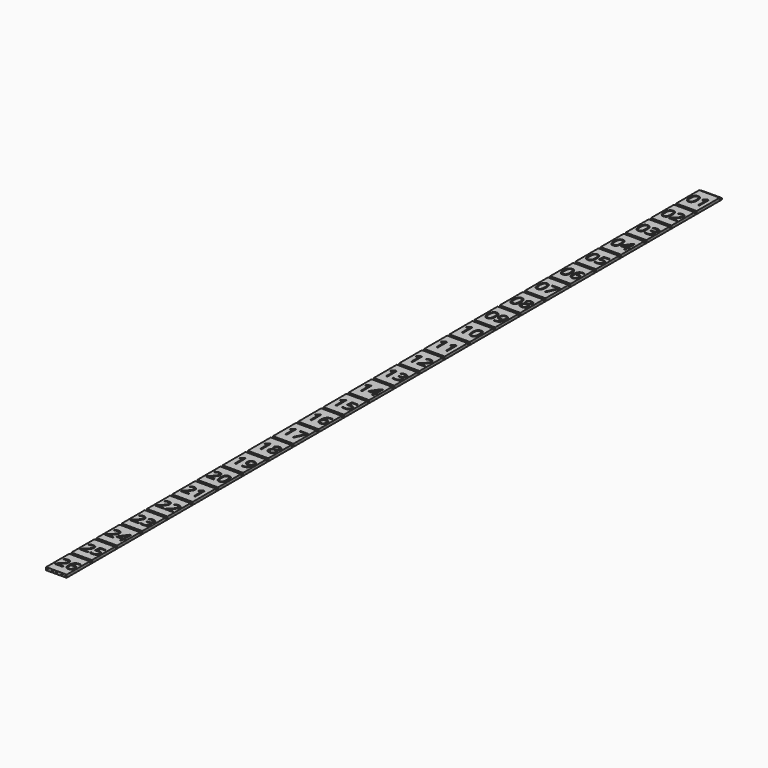
from build123d import *

# Parameters (mm, degrees)
F0_W     = 5.9
F0_H     = 8.26
F1_DEPTH = 0.4
F2_DEPTH = 0.4
F4_DEPTH = 0.4


with BuildPart() as f1:
    # F0 (on Top) → F1 (new body)
    with BuildSketch(Plane.XY):
        with Locations((3.75, -4.93)):
            Rectangle(F0_W, F0_H)
        with BuildLine():
            add(Edge.make_bspline(
                [(3.3188151042, -3.6283702257), (3.6086501736, -4.0815190972), (3.6086501736, -4.9397612847)],
                knots=[0, 0, 0, 1, 1, 1], degree=2))
            add(Edge.make_bspline(
                [(3.6086501736, -4.9397612847), (3.6086501736, -5.8295399306), (3.3282009549, -6.268422309)],
                knots=[0, 0, 0, 1, 1, 1], degree=2))
            add(Edge.make_bspline(
                [(3.3282009549, -6.268422309), (3.0477517361, -6.7073046875), (2.4703342014, -6.7073046875)],
                knots=[0, 0, 0, 1, 1, 1], degree=2))
            add(Edge.make_bspline(
                [(2.4703342014, -6.7073046875), (1.9169444444, -6.7073046875), (1.6282356771, -6.2579101563)],
                knots=[0, 0, 0, 1, 1, 1], degree=2))
            add(Edge.make_bspline(
                [(1.6282356771, -6.2579101563), (1.3395269097, -5.808515625), (1.3395269097, -4.9397612847)],
                knots=[0, 0, 0, 1, 1, 1], degree=2))
            add(Edge.make_bspline(
                [(1.3395269097, -4.9397612847), (1.3395269097, -4.0439756944), (1.6188498264, -3.6095985243)],
                knots=[0, 0, 0, 1, 1, 1], degree=2))
            add(Edge.make_bspline(
                [(1.6188498264, -3.6095985243), (1.8981727431, -3.1752213542), (2.4703342014, -3.1752213542)],
                knots=[0, 0, 0, 1, 1, 1], degree=2))
            add(Edge.make_bspline(
                [(2.4703342014, -3.1752213542), (3.0289800347, -3.1752213542), (3.3188151042, -3.6283702257)],
                knots=[0, 0, 0, 1, 1, 1], degree=2))
        make_face(mode=Mode.SUBTRACT)
        with BuildLine():
            Line((5.5248654514, -3.2292838542), (5.5248654514, -6.66))
            Line((5.5248654514, -6.66), (5.1449262153, -6.66))
            Line((5.1449262153, -6.66), (5.1449262153, -4.2151736111))
            add(Edge.make_bspline(
                [(5.1449262153, -4.2151736111), (5.1449262153, -3.9095703125), (5.1636979167, -3.6377560764)],
                knots=[0, 0, 0, 1, 1, 1], degree=2))
            add(Edge.make_bspline(
                [(5.1636979167, -3.6377560764), (5.1148914931, -3.6873133681), (5.0536957465, -3.741000434)],
                knots=[0, 0, 0, 1, 1, 1], degree=2))
            add(Edge.make_bspline(
                [(5.0536957465, -3.741000434), (4.9925, -3.7946875), (4.4954253472, -4.1986545139)],
                knots=[0, 0, 0, 1, 1, 1], degree=2))
            Line((4.4954253472, -4.1986545139), (4.2889366319, -3.9313454861))
            Line((4.2889366319, -3.9313454861), (5.1967361111, -3.2292838542))
            Line((5.1967361111, -3.2292838542), (5.5248654514, -3.2292838542))
        make_face(mode=Mode.SUBTRACT)
    extrude(amount=F1_DEPTH)


with BuildPart() as f2:
    # F0 (on Top) → F2 (new body)
    with BuildSketch(Plane.XY):
        with BuildLine():
            add(Edge.make_bspline(
                [(1.9098111979, -3.8521289062), (1.7337326389, -4.1911458333), (1.7337326389, -4.9397612847)],
                knots=[0, 0, 0, 1, 1, 1], degree=2))
            add(Edge.make_bspline(
                [(1.7337326389, -4.9397612847), (1.7337326389, -5.6883767361), (1.9098111979, -6.0300217014)],
                knots=[0, 0, 0, 1, 1, 1], degree=2))
            add(Edge.make_bspline(
                [(1.9098111979, -6.0300217014), (2.0858897569, -6.3716666667), (2.4703342014, -6.3716666667)],
                knots=[0, 0, 0, 1, 1, 1], degree=2))
            add(Edge.make_bspline(
                [(2.4703342014, -6.3716666667), (2.8600347222, -6.3716666667), (3.0346115451, -6.0255164931)],
                knots=[0, 0, 0, 1, 1, 1], degree=2))
            add(Edge.make_bspline(
                [(3.0346115451, -6.0255164931), (3.2091883681, -5.6793663194), (3.2091883681, -4.9397612847)],
                knots=[0, 0, 0, 1, 1, 1], degree=2))
            add(Edge.make_bspline(
                [(3.2091883681, -4.9397612847), (3.2091883681, -4.2009071181), (3.0346115451, -3.8570095486)],
                knots=[0, 0, 0, 1, 1, 1], degree=2))
            add(Edge.make_bspline(
                [(3.0346115451, -3.8570095486), (2.8600347222, -3.5131119792), (2.4703342014, -3.5131119792)],
                knots=[0, 0, 0, 1, 1, 1], degree=2))
            add(Edge.make_bspline(
                [(2.4703342014, -3.5131119792), (2.0858897569, -3.5131119792), (1.9098111979, -3.8521289062)],
                knots=[0, 0, 0, 1, 1, 1], degree=2))
        make_face()
    extrude(amount=F2_DEPTH)


with BuildPart() as f2b:
    # F0 (on Top) → F2, piece 2 (new body)
    with BuildSketch(Plane.XY):
        with Locations((3.75, -13.99)):
            Rectangle(F0_W, F0_H)
        with BuildLine():
            add(Edge.make_bspline(
                [(3.3188151042, -12.6883702257), (3.6086501736, -13.1415190972), (3.6086501736, -13.9997612847)],
                knots=[0, 0, 0, 1, 1, 1], degree=2))
            add(Edge.make_bspline(
                [(3.6086501736, -13.9997612847), (3.6086501736, -14.8895399306), (3.3282009549, -15.328422309)],
                knots=[0, 0, 0, 1, 1, 1], degree=2))
            add(Edge.make_bspline(
                [(3.3282009549, -15.328422309), (3.0477517361, -15.7673046875), (2.4703342014, -15.7673046875)],
                knots=[0, 0, 0, 1, 1, 1], degree=2))
            add(Edge.make_bspline(
                [(2.4703342014, -15.7673046875), (1.9169444444, -15.7673046875), (1.6282356771, -15.3179101562)],
                knots=[0, 0, 0, 1, 1, 1], degree=2))
            add(Edge.make_bspline(
                [(1.6282356771, -15.3179101562), (1.3395269097, -14.868515625), (1.3395269097, -13.9997612847)],
                knots=[0, 0, 0, 1, 1, 1], degree=2))
            add(Edge.make_bspline(
                [(1.3395269097, -13.9997612847), (1.3395269097, -13.1039756944), (1.6188498264, -12.6695985243)],
                knots=[0, 0, 0, 1, 1, 1], degree=2))
            add(Edge.make_bspline(
                [(1.6188498264, -12.6695985243), (1.8981727431, -12.2352213542), (2.4703342014, -12.2352213542)],
                knots=[0, 0, 0, 1, 1, 1], degree=2))
            add(Edge.make_bspline(
                [(2.4703342014, -12.2352213542), (3.0289800347, -12.2352213542), (3.3188151042, -12.6883702257)],
                knots=[0, 0, 0, 1, 1, 1], degree=2))
        make_face(mode=Mode.SUBTRACT)
        with BuildLine():
            Line((6.3373046875, -15.3588324653), (6.3373046875, -15.72))
            Line((6.3373046875, -15.72), (4.0824479167, -15.72))
            Line((4.0824479167, -15.72), (4.0824479167, -15.3843619792))
            Line((4.0824479167, -15.3843619792), (4.9857421875, -14.4765625))
            add(Edge.make_bspline(
                [(4.9857421875, -14.4765625), (5.3987196181, -14.0583289931), (5.5301215278, -13.8799978299)],
                knots=[0, 0, 0, 1, 1, 1], degree=2))
            add(Edge.make_bspline(
                [(5.5301215278, -13.8799978299), (5.6615234375, -13.7016666667), (5.7272243924, -13.5327213542)],
                knots=[0, 0, 0, 1, 1, 1], degree=2))
            add(Edge.make_bspline(
                [(5.7272243924, -13.5327213542), (5.7929253472, -13.3637760417), (5.7929253472, -13.1693012153)],
                knots=[0, 0, 0, 1, 1, 1], degree=2))
            add(Edge.make_bspline(
                [(5.7929253472, -13.1693012153), (5.7929253472, -12.8944835069), (5.6262326389, -12.7337977431)],
                knots=[0, 0, 0, 1, 1, 1], degree=2))
            add(Edge.make_bspline(
                [(5.6262326389, -12.7337977431), (5.4595399306, -12.5731119792), (5.1636979167, -12.5731119792)],
                knots=[0, 0, 0, 1, 1, 1], degree=2))
            add(Edge.make_bspline(
                [(5.1636979167, -12.5731119792), (4.9504513889, -12.5731119792), (4.7589800347, -12.6436935764)],
                knots=[0, 0, 0, 1, 1, 1], degree=2))
            add(Edge.make_bspline(
                [(4.7589800347, -12.6436935764), (4.5675086806, -12.7142751736), (4.3332378472, -12.8997395833)],
                knots=[0, 0, 0, 1, 1, 1], degree=2))
            Line((4.3332378472, -12.8997395833), (4.1267491319, -12.6346831597))
            add(Edge.make_bspline(
                [(4.1267491319, -12.6346831597), (4.600546875, -12.2404774306), (5.1591927083, -12.2404774306)],
                knots=[0, 0, 0, 1, 1, 1], degree=2))
            add(Edge.make_bspline(
                [(5.1591927083, -12.2404774306), (5.6427517361, -12.2404774306), (5.9171940104, -12.4878884549)],
                knots=[0, 0, 0, 1, 1, 1], degree=2))
            add(Edge.make_bspline(
                [(5.9171940104, -12.4878884549), (6.1916362847, -12.7352994792), (6.1916362847, -13.1527821181)],
                knots=[0, 0, 0, 1, 1, 1], degree=2))
            add(Edge.make_bspline(
                [(6.1916362847, -13.1527821181), (6.1916362847, -13.4794097222), (6.0084244792, -13.7985286458)],
                knots=[0, 0, 0, 1, 1, 1], degree=2))
            add(Edge.make_bspline(
                [(6.0084244792, -13.7985286458), (5.8252126736, -14.1176475694), (5.3236328125, -14.6057118056)],
                knots=[0, 0, 0, 1, 1, 1], degree=2))
            Line((5.3236328125, -14.6057118056), (4.5727647569, -15.3400607639))
            Line((4.5727647569, -15.3400607639), (4.5727647569, -15.3588324653))
            Line((4.5727647569, -15.3588324653), (6.3373046875, -15.3588324653))
        make_face(mode=Mode.SUBTRACT)
    extrude(amount=F2_DEPTH)


with BuildPart() as f2c:
    # F0 (on Top) → F2, piece 3 (new body)
    with BuildSketch(Plane.XY):
        with BuildLine():
            add(Edge.make_bspline(
                [(1.9098111979, -12.9121289062), (1.7337326389, -13.2511458333), (1.7337326389, -13.9997612847)],
                knots=[0, 0, 0, 1, 1, 1], degree=2))
            add(Edge.make_bspline(
                [(1.7337326389, -13.9997612847), (1.7337326389, -14.7483767361), (1.9098111979, -15.0900217014)],
                knots=[0, 0, 0, 1, 1, 1], degree=2))
            add(Edge.make_bspline(
                [(1.9098111979, -15.0900217014), (2.0858897569, -15.4316666667), (2.4703342014, -15.4316666667)],
                knots=[0, 0, 0, 1, 1, 1], degree=2))
            add(Edge.make_bspline(
                [(2.4703342014, -15.4316666667), (2.8600347222, -15.4316666667), (3.0346115451, -15.0855164931)],
                knots=[0, 0, 0, 1, 1, 1], degree=2))
            add(Edge.make_bspline(
                [(3.0346115451, -15.0855164931), (3.2091883681, -14.7393663194), (3.2091883681, -13.9997612847)],
                knots=[0, 0, 0, 1, 1, 1], degree=2))
            add(Edge.make_bspline(
                [(3.2091883681, -13.9997612847), (3.2091883681, -13.2609071181), (3.0346115451, -12.9170095486)],
                knots=[0, 0, 0, 1, 1, 1], degree=2))
            add(Edge.make_bspline(
                [(3.0346115451, -12.9170095486), (2.8600347222, -12.5731119792), (2.4703342014, -12.5731119792)],
                knots=[0, 0, 0, 1, 1, 1], degree=2))
            add(Edge.make_bspline(
                [(2.4703342014, -12.5731119792), (2.0858897569, -12.5731119792), (1.9098111979, -12.9121289062)],
                knots=[0, 0, 0, 1, 1, 1], degree=2))
        make_face()
    extrude(amount=F2_DEPTH)


with BuildPart() as f2d:
    # F0 (on Top) → F2, piece 4 (new body)
    with BuildSketch(Plane.XY):
        with Locations((3.75, -23.05)):
            Rectangle(F0_W, F0_H)
        with BuildLine():
            add(Edge.make_bspline(
                [(3.3188151042, -21.7483702257), (3.6086501736, -22.2015190972), (3.6086501736, -23.0597612847)],
                knots=[0, 0, 0, 1, 1, 1], degree=2))
            add(Edge.make_bspline(
                [(3.6086501736, -23.0597612847), (3.6086501736, -23.9495399306), (3.3282009549, -24.388422309)],
                knots=[0, 0, 0, 1, 1, 1], degree=2))
            add(Edge.make_bspline(
                [(3.3282009549, -24.388422309), (3.0477517361, -24.8273046875), (2.4703342014, -24.8273046875)],
                knots=[0, 0, 0, 1, 1, 1], degree=2))
            add(Edge.make_bspline(
                [(2.4703342014, -24.8273046875), (1.9169444444, -24.8273046875), (1.6282356771, -24.3779101562)],
                knots=[0, 0, 0, 1, 1, 1], degree=2))
            add(Edge.make_bspline(
                [(1.6282356771, -24.3779101562), (1.3395269097, -23.928515625), (1.3395269097, -23.0597612847)],
                knots=[0, 0, 0, 1, 1, 1], degree=2))
            add(Edge.make_bspline(
                [(1.3395269097, -23.0597612847), (1.3395269097, -22.1639756944), (1.6188498264, -21.7295985243)],
                knots=[0, 0, 0, 1, 1, 1], degree=2))
            add(Edge.make_bspline(
                [(1.6188498264, -21.7295985243), (1.8981727431, -21.2952213542), (2.4703342014, -21.2952213542)],
                knots=[0, 0, 0, 1, 1, 1], degree=2))
            add(Edge.make_bspline(
                [(2.4703342014, -21.2952213542), (3.0289800347, -21.2952213542), (3.3188151042, -21.7483702257)],
                knots=[0, 0, 0, 1, 1, 1], degree=2))
        make_face(mode=Mode.SUBTRACT)
        with BuildLine():
            add(Edge.make_bspline(
                [(5.9310850694, -21.5291167535), (6.2081553819, -21.7577560764), (6.2081553819, -22.1564670139)],
                knots=[0, 0, 0, 1, 1, 1], degree=2))
            add(Edge.make_bspline(
                [(6.2081553819, -22.1564670139), (6.2081553819, -22.4853472222), (6.0238172743, -22.6940885417)],
                knots=[0, 0, 0, 1, 1, 1], degree=2))
            add(Edge.make_bspline(
                [(6.0238172743, -22.6940885417), (5.8394791667, -22.9028298611), (5.5015885417, -22.9734114583)],
                knots=[0, 0, 0, 1, 1, 1], degree=2))
            Line((5.5015885417, -22.9734114583), (5.5015885417, -22.9921831597))
            add(Edge.make_bspline(
                [(5.5015885417, -22.9921831597), (5.9145659722, -23.0432421875), (6.113921441, -23.2546115451)],
                knots=[0, 0, 0, 1, 1, 1], degree=2))
            add(Edge.make_bspline(
                [(6.113921441, -23.2546115451), (6.3132769097, -23.4659809028), (6.3132769097, -23.8083767361)],
                knots=[0, 0, 0, 1, 1, 1], degree=2))
            add(Edge.make_bspline(
                [(6.3132769097, -23.8083767361), (6.3132769097, -24.2986935764), (5.9731336806, -24.5629991319)],
                knots=[0, 0, 0, 1, 1, 1], degree=2))
            add(Edge.make_bspline(
                [(5.9731336806, -24.5629991319), (5.6329904514, -24.8273046875), (5.0067664931, -24.8273046875)],
                knots=[0, 0, 0, 1, 1, 1], degree=2))
            add(Edge.make_bspline(
                [(5.0067664931, -24.8273046875), (4.7342013889, -24.8273046875), (4.5078146701, -24.7860069444)],
                knots=[0, 0, 0, 1, 1, 1], degree=2))
            add(Edge.make_bspline(
                [(4.5078146701, -24.7860069444), (4.2814279514, -24.7447092014), (4.0681814236, -24.6418402778)],
                knots=[0, 0, 0, 1, 1, 1], degree=2))
            Line((4.0681814236, -24.6418402778), (4.0681814236, -24.2709114583))
            add(Edge.make_bspline(
                [(4.0681814236, -24.2709114583), (4.2911892361, -24.3812890625), (4.5434809028, -24.4387304687)],
                knots=[0, 0, 0, 1, 1, 1], degree=2))
            add(Edge.make_bspline(
                [(4.5434809028, -24.4387304687), (4.7957725694, -24.496171875), (5.0210329861, -24.496171875)],
                knots=[0, 0, 0, 1, 1, 1], degree=2))
            add(Edge.make_bspline(
                [(5.0210329861, -24.496171875), (5.9100607639, -24.496171875), (5.9100607639, -23.7993663194)],
                knots=[0, 0, 0, 1, 1, 1], degree=2))
            add(Edge.make_bspline(
                [(5.9100607639, -23.7993663194), (5.9100607639, -23.1746440972), (4.9294270833, -23.1746440972)],
                knots=[0, 0, 0, 1, 1, 1], degree=2))
            Line((4.9294270833, -23.1746440972), (4.5915364583, -23.1746440972))
            Line((4.5915364583, -23.1746440972), (4.5915364583, -22.8397569444))
            Line((4.5915364583, -22.8397569444), (4.9339322917, -22.8397569444))
            add(Edge.make_bspline(
                [(4.9339322917, -22.8397569444), (5.3348958333, -22.8397569444), (5.5695421007, -22.6625520833)],
                knots=[0, 0, 0, 1, 1, 1], degree=2))
            add(Edge.make_bspline(
                [(5.5695421007, -22.6625520833), (5.8041883681, -22.4853472222), (5.8041883681, -22.1707335069)],
                knots=[0, 0, 0, 1, 1, 1], degree=2))
            add(Edge.make_bspline(
                [(5.8041883681, -22.1707335069), (5.8041883681, -21.9199435764), (5.6318641493, -21.7765277778)],
                knots=[0, 0, 0, 1, 1, 1], degree=2))
            add(Edge.make_bspline(
                [(5.6318641493, -21.7765277778), (5.4595399306, -21.6331119792), (5.1636979167, -21.6331119792)],
                knots=[0, 0, 0, 1, 1, 1], degree=2))
            add(Edge.make_bspline(
                [(5.1636979167, -21.6331119792), (4.9384375, -21.6331119792), (4.7390820312, -21.6943077257)],
                knots=[0, 0, 0, 1, 1, 1], degree=2))
            add(Edge.make_bspline(
                [(4.7390820312, -21.6943077257), (4.5397265625, -21.7555034722), (4.2836805556, -21.9199435764)],
                knots=[0, 0, 0, 1, 1, 1], degree=2))
            Line((4.2836805556, -21.9199435764), (4.086953125, -21.6571397569))
            add(Edge.make_bspline(
                [(4.086953125, -21.6571397569), (4.2979470486, -21.4904470486), (4.573515625, -21.3954622396)],
                knots=[0, 0, 0, 1, 1, 1], degree=2))
            add(Edge.make_bspline(
                [(4.573515625, -21.3954622396), (4.8490842014, -21.3004774306), (5.1546875, -21.3004774306)],
                knots=[0, 0, 0, 1, 1, 1], degree=2))
            add(Edge.make_bspline(
                [(5.1546875, -21.3004774306), (5.6540147569, -21.3004774306), (5.9310850694, -21.5291167535)],
                knots=[0, 0, 0, 1, 1, 1], degree=2))
        make_face(mode=Mode.SUBTRACT)
    extrude(amount=F2_DEPTH)


with BuildPart() as f2e:
    # F0 (on Top) → F2, piece 5 (new body)
    with BuildSketch(Plane.XY):
        with BuildLine():
            add(Edge.make_bspline(
                [(1.9098111979, -21.9721289062), (1.7337326389, -22.3111458333), (1.7337326389, -23.0597612847)],
                knots=[0, 0, 0, 1, 1, 1], degree=2))
            add(Edge.make_bspline(
                [(1.7337326389, -23.0597612847), (1.7337326389, -23.8083767361), (1.9098111979, -24.1500217014)],
                knots=[0, 0, 0, 1, 1, 1], degree=2))
            add(Edge.make_bspline(
                [(1.9098111979, -24.1500217014), (2.0858897569, -24.4916666667), (2.4703342014, -24.4916666667)],
                knots=[0, 0, 0, 1, 1, 1], degree=2))
            add(Edge.make_bspline(
                [(2.4703342014, -24.4916666667), (2.8600347222, -24.4916666667), (3.0346115451, -24.1455164931)],
                knots=[0, 0, 0, 1, 1, 1], degree=2))
            add(Edge.make_bspline(
                [(3.0346115451, -24.1455164931), (3.2091883681, -23.7993663194), (3.2091883681, -23.0597612847)],
                knots=[0, 0, 0, 1, 1, 1], degree=2))
            add(Edge.make_bspline(
                [(3.2091883681, -23.0597612847), (3.2091883681, -22.3209071181), (3.0346115451, -21.9770095486)],
                knots=[0, 0, 0, 1, 1, 1], degree=2))
            add(Edge.make_bspline(
                [(3.0346115451, -21.9770095486), (2.8600347222, -21.6331119792), (2.4703342014, -21.6331119792)],
                knots=[0, 0, 0, 1, 1, 1], degree=2))
            add(Edge.make_bspline(
                [(2.4703342014, -21.6331119792), (2.0858897569, -21.6331119792), (1.9098111979, -21.9721289062)],
                knots=[0, 0, 0, 1, 1, 1], degree=2))
        make_face()
    extrude(amount=F2_DEPTH)


with BuildPart() as f2f:
    # F0 (on Top) → F2, piece 6 (new body)
    with BuildSketch(Plane.XY):
        with Locations((3.75, -32.11)):
            Rectangle(F0_W, F0_H)
        with BuildLine():
            add(Edge.make_bspline(
                [(3.3188151042, -30.8083702257), (3.6086501736, -31.2615190972), (3.6086501736, -32.1197612847)],
                knots=[0, 0, 0, 1, 1, 1], degree=2))
            add(Edge.make_bspline(
                [(3.6086501736, -32.1197612847), (3.6086501736, -33.0095399306), (3.3282009549, -33.448422309)],
                knots=[0, 0, 0, 1, 1, 1], degree=2))
            add(Edge.make_bspline(
                [(3.3282009549, -33.448422309), (3.0477517361, -33.8873046875), (2.4703342014, -33.8873046875)],
                knots=[0, 0, 0, 1, 1, 1], degree=2))
            add(Edge.make_bspline(
                [(2.4703342014, -33.8873046875), (1.9169444444, -33.8873046875), (1.6282356771, -33.4379101562)],
                knots=[0, 0, 0, 1, 1, 1], degree=2))
            add(Edge.make_bspline(
                [(1.6282356771, -33.4379101562), (1.3395269097, -32.988515625), (1.3395269097, -32.1197612847)],
                knots=[0, 0, 0, 1, 1, 1], degree=2))
            add(Edge.make_bspline(
                [(1.3395269097, -32.1197612847), (1.3395269097, -31.2239756944), (1.6188498264, -30.7895985243)],
                knots=[0, 0, 0, 1, 1, 1], degree=2))
            add(Edge.make_bspline(
                [(1.6188498264, -30.7895985243), (1.8981727431, -30.3552213542), (2.4703342014, -30.3552213542)],
                knots=[0, 0, 0, 1, 1, 1], degree=2))
            add(Edge.make_bspline(
                [(2.4703342014, -30.3552213542), (3.0289800347, -30.3552213542), (3.3188151042, -30.8083702257)],
                knots=[0, 0, 0, 1, 1, 1], degree=2))
        make_face(mode=Mode.SUBTRACT)
        Polygon((6.4987413194, -32.6971788194), (6.4987413194, -33.0515885417), (5.9896527778, -33.0515885417), (5.9896527778, -33.84), (5.6164713542, -33.84), (5.6164713542, -33.0515885417), (3.9480425347, -33.0515885417), (3.9480425347, -32.7114453125), (5.5766753472, -30.3905121528), (5.9896527778, -30.3905121528), (5.9896527778, -32.6971788194), align=None, mode=Mode.SUBTRACT)
    extrude(amount=F2_DEPTH)


with BuildPart() as f2g:
    # F0 (on Top) → F2, piece 7 (new body)
    with BuildSketch(Plane.XY):
        with BuildLine():
            add(Edge.make_bspline(
                [(1.9098111979, -31.0321289062), (1.7337326389, -31.3711458333), (1.7337326389, -32.1197612847)],
                knots=[0, 0, 0, 1, 1, 1], degree=2))
            add(Edge.make_bspline(
                [(1.7337326389, -32.1197612847), (1.7337326389, -32.8683767361), (1.9098111979, -33.2100217014)],
                knots=[0, 0, 0, 1, 1, 1], degree=2))
            add(Edge.make_bspline(
                [(1.9098111979, -33.2100217014), (2.0858897569, -33.5516666667), (2.4703342014, -33.5516666667)],
                knots=[0, 0, 0, 1, 1, 1], degree=2))
            add(Edge.make_bspline(
                [(2.4703342014, -33.5516666667), (2.8600347222, -33.5516666667), (3.0346115451, -33.2055164931)],
                knots=[0, 0, 0, 1, 1, 1], degree=2))
            add(Edge.make_bspline(
                [(3.0346115451, -33.2055164931), (3.2091883681, -32.8593663194), (3.2091883681, -32.1197612847)],
                knots=[0, 0, 0, 1, 1, 1], degree=2))
            add(Edge.make_bspline(
                [(3.2091883681, -32.1197612847), (3.2091883681, -31.3809071181), (3.0346115451, -31.0370095486)],
                knots=[0, 0, 0, 1, 1, 1], degree=2))
            add(Edge.make_bspline(
                [(3.0346115451, -31.0370095486), (2.8600347222, -30.6931119792), (2.4703342014, -30.6931119792)],
                knots=[0, 0, 0, 1, 1, 1], degree=2))
            add(Edge.make_bspline(
                [(2.4703342014, -30.6931119792), (2.0858897569, -30.6931119792), (1.9098111979, -31.0321289062)],
                knots=[0, 0, 0, 1, 1, 1], degree=2))
        make_face()
    extrude(amount=F2_DEPTH)


with BuildPart() as f2h:
    # F0 (on Top) → F2, piece 8 (new body)
    with BuildSketch(Plane.XY):
        with BuildLine():
            Line((4.3377430556, -32.6971788194), (5.6164713542, -32.6971788194))
            Line((5.6164713542, -32.6971788194), (5.6164713542, -31.5566102431))
            add(Edge.make_bspline(
                [(5.6164713542, -31.5566102431), (5.6164713542, -31.2209722222), (5.6404991319, -30.798984375)],
                knots=[0, 0, 0, 1, 1, 1], degree=2))
            Line((5.6404991319, -30.798984375), (5.6217274306, -30.798984375))
            add(Edge.make_bspline(
                [(5.6217274306, -30.798984375), (5.5090972222, -31.0242447917), (5.4099826389, -31.1721657986)],
                knots=[0, 0, 0, 1, 1, 1], degree=2))
            Line((5.4099826389, -31.1721657986), (4.3377430556, -32.6971788194))
        make_face()
    extrude(amount=F2_DEPTH)


with BuildPart() as f2i:
    # F0 (on Top) → F2, piece 9 (new body)
    with BuildSketch(Plane.XY):
        with Locations((3.75, -41.17)):
            Rectangle(F0_W, F0_H)
        with BuildLine():
            add(Edge.make_bspline(
                [(3.3188151042, -39.8683702257), (3.6086501736, -40.3215190972), (3.6086501736, -41.1797612847)],
                knots=[0, 0, 0, 1, 1, 1], degree=2))
            add(Edge.make_bspline(
                [(3.6086501736, -41.1797612847), (3.6086501736, -42.0695399306), (3.3282009549, -42.508422309)],
                knots=[0, 0, 0, 1, 1, 1], degree=2))
            add(Edge.make_bspline(
                [(3.3282009549, -42.508422309), (3.0477517361, -42.9473046875), (2.4703342014, -42.9473046875)],
                knots=[0, 0, 0, 1, 1, 1], degree=2))
            add(Edge.make_bspline(
                [(2.4703342014, -42.9473046875), (1.9169444444, -42.9473046875), (1.6282356771, -42.4979101562)],
                knots=[0, 0, 0, 1, 1, 1], degree=2))
            add(Edge.make_bspline(
                [(1.6282356771, -42.4979101562), (1.3395269097, -42.048515625), (1.3395269097, -41.1797612847)],
                knots=[0, 0, 0, 1, 1, 1], degree=2))
            add(Edge.make_bspline(
                [(1.3395269097, -41.1797612847), (1.3395269097, -40.2839756944), (1.6188498264, -39.8495985243)],
                knots=[0, 0, 0, 1, 1, 1], degree=2))
            add(Edge.make_bspline(
                [(1.6188498264, -39.8495985243), (1.8981727431, -39.4152213542), (2.4703342014, -39.4152213542)],
                knots=[0, 0, 0, 1, 1, 1], degree=2))
            add(Edge.make_bspline(
                [(2.4703342014, -39.4152213542), (3.0289800347, -39.4152213542), (3.3188151042, -39.8683702257)],
                knots=[0, 0, 0, 1, 1, 1], degree=2))
        make_face(mode=Mode.SUBTRACT)
        with BuildLine():
            add(Edge.make_bspline(
                [(4.6170659722, -40.8583897569), (4.8866276042, -40.8043272569), (5.1546875, -40.8043272569)],
                knots=[0, 0, 0, 1, 1, 1], degree=2))
            add(Edge.make_bspline(
                [(5.1546875, -40.8043272569), (5.6968142361, -40.8043272569), (6.0076736111, -41.0731380208)],
                knots=[0, 0, 0, 1, 1, 1], degree=2))
            add(Edge.make_bspline(
                [(6.0076736111, -41.0731380208), (6.3185329861, -41.3419487847), (6.3185329861, -41.8089887153)],
                knots=[0, 0, 0, 1, 1, 1], degree=2))
            add(Edge.make_bspline(
                [(6.3185329861, -41.8089887153), (6.3185329861, -42.3413541667), (5.979516059, -42.6443294271)],
                knots=[0, 0, 0, 1, 1, 1], degree=2))
            add(Edge.make_bspline(
                [(5.979516059, -42.6443294271), (5.6404991319, -42.9473046875), (5.0443098958, -42.9473046875)],
                knots=[0, 0, 0, 1, 1, 1], degree=2))
            add(Edge.make_bspline(
                [(5.0443098958, -42.9473046875), (4.4646397569, -42.9473046875), (4.1597873264, -42.7618402778)],
                knots=[0, 0, 0, 1, 1, 1], degree=2))
            Line((4.1597873264, -42.7618402778), (4.1597873264, -42.38640625))
            add(Edge.make_bspline(
                [(4.1597873264, -42.38640625), (4.3234765625, -42.4915277778), (4.5675086806, -42.5515972222)],
                knots=[0, 0, 0, 1, 1, 1], degree=2))
            add(Edge.make_bspline(
                [(4.5675086806, -42.5515972222), (4.8115407986, -42.6116666667), (5.0488151042, -42.6116666667)],
                knots=[0, 0, 0, 1, 1, 1], degree=2))
            add(Edge.make_bspline(
                [(5.0488151042, -42.6116666667), (5.4617925347, -42.6116666667), (5.6904318576, -42.4168164062)],
                knots=[0, 0, 0, 1, 1, 1], degree=2))
            add(Edge.make_bspline(
                [(5.6904318576, -42.4168164062), (5.9190711806, -42.2219661458), (5.9190711806, -41.8532899306)],
                knots=[0, 0, 0, 1, 1, 1], degree=2))
            add(Edge.make_bspline(
                [(5.9190711806, -41.8532899306), (5.9190711806, -41.1354600694), (5.0398046875, -41.1354600694)],
                knots=[0, 0, 0, 1, 1, 1], degree=2))
            add(Edge.make_bspline(
                [(5.0398046875, -41.1354600694), (4.816796875, -41.1354600694), (4.4436154514, -41.2037890625)],
                knots=[0, 0, 0, 1, 1, 1], degree=2))
            Line((4.4436154514, -41.2037890625), (4.2416319444, -41.0746397569))
            Line((4.2416319444, -41.0746397569), (4.37078125, -39.4692838542))
            Line((4.37078125, -39.4692838542), (6.0767534722, -39.4692838542))
            Line((6.0767534722, -39.4692838542), (6.0767534722, -39.8281987847))
            Line((6.0767534722, -39.8281987847), (4.7041666667, -39.8281987847))
            Line((4.7041666667, -39.8281987847), (4.6170659722, -40.8583897569))
        make_face(mode=Mode.SUBTRACT)
    extrude(amount=F2_DEPTH)


with BuildPart() as f2j:
    # F0 (on Top) → F2, piece 10 (new body)
    with BuildSketch(Plane.XY):
        with BuildLine():
            add(Edge.make_bspline(
                [(1.9098111979, -40.0921289062), (1.7337326389, -40.4311458333), (1.7337326389, -41.1797612847)],
                knots=[0, 0, 0, 1, 1, 1], degree=2))
            add(Edge.make_bspline(
                [(1.7337326389, -41.1797612847), (1.7337326389, -41.9283767361), (1.9098111979, -42.2700217014)],
                knots=[0, 0, 0, 1, 1, 1], degree=2))
            add(Edge.make_bspline(
                [(1.9098111979, -42.2700217014), (2.0858897569, -42.6116666667), (2.4703342014, -42.6116666667)],
                knots=[0, 0, 0, 1, 1, 1], degree=2))
            add(Edge.make_bspline(
                [(2.4703342014, -42.6116666667), (2.8600347222, -42.6116666667), (3.0346115451, -42.2655164931)],
                knots=[0, 0, 0, 1, 1, 1], degree=2))
            add(Edge.make_bspline(
                [(3.0346115451, -42.2655164931), (3.2091883681, -41.9193663194), (3.2091883681, -41.1797612847)],
                knots=[0, 0, 0, 1, 1, 1], degree=2))
            add(Edge.make_bspline(
                [(3.2091883681, -41.1797612847), (3.2091883681, -40.4409071181), (3.0346115451, -40.0970095486)],
                knots=[0, 0, 0, 1, 1, 1], degree=2))
            add(Edge.make_bspline(
                [(3.0346115451, -40.0970095486), (2.8600347222, -39.7531119792), (2.4703342014, -39.7531119792)],
                knots=[0, 0, 0, 1, 1, 1], degree=2))
            add(Edge.make_bspline(
                [(2.4703342014, -39.7531119792), (2.0858897569, -39.7531119792), (1.9098111979, -40.0921289062)],
                knots=[0, 0, 0, 1, 1, 1], degree=2))
        make_face()
    extrude(amount=F2_DEPTH)


with BuildPart() as f2k:
    # F0 (on Top) → F2, piece 11 (new body)
    with BuildSketch(Plane.XY):
        with Locations((3.75, -50.23)):
            Rectangle(F0_W, F0_H)
        with BuildLine():
            add(Edge.make_bspline(
                [(3.3188151042, -48.9283702257), (3.6086501736, -49.3815190972), (3.6086501736, -50.2397612847)],
                knots=[0, 0, 0, 1, 1, 1], degree=2))
            add(Edge.make_bspline(
                [(3.6086501736, -50.2397612847), (3.6086501736, -51.1295399306), (3.3282009549, -51.568422309)],
                knots=[0, 0, 0, 1, 1, 1], degree=2))
            add(Edge.make_bspline(
                [(3.3282009549, -51.568422309), (3.0477517361, -52.0073046875), (2.4703342014, -52.0073046875)],
                knots=[0, 0, 0, 1, 1, 1], degree=2))
            add(Edge.make_bspline(
                [(2.4703342014, -52.0073046875), (1.9169444444, -52.0073046875), (1.6282356771, -51.5579101562)],
                knots=[0, 0, 0, 1, 1, 1], degree=2))
            add(Edge.make_bspline(
                [(1.6282356771, -51.5579101562), (1.3395269097, -51.108515625), (1.3395269097, -50.2397612847)],
                knots=[0, 0, 0, 1, 1, 1], degree=2))
            add(Edge.make_bspline(
                [(1.3395269097, -50.2397612847), (1.3395269097, -49.3439756944), (1.6188498264, -48.9095985243)],
                knots=[0, 0, 0, 1, 1, 1], degree=2))
            add(Edge.make_bspline(
                [(1.6188498264, -48.9095985243), (1.8981727431, -48.4752213542), (2.4703342014, -48.4752213542)],
                knots=[0, 0, 0, 1, 1, 1], degree=2))
            add(Edge.make_bspline(
                [(2.4703342014, -48.4752213542), (3.0289800347, -48.4752213542), (3.3188151042, -48.9283702257)],
                knots=[0, 0, 0, 1, 1, 1], degree=2))
        make_face(mode=Mode.SUBTRACT)
        with BuildLine():
            add(Edge.make_bspline(
                [(4.4342296007, -51.6070920139), (4.1222439236, -51.2068793403), (4.1222439236, -50.4935546875)],
                knots=[0, 0, 0, 1, 1, 1], degree=2))
            add(Edge.make_bspline(
                [(4.1222439236, -50.4935546875), (4.1222439236, -49.4821354167), (4.5153233507, -48.9813064236)],
                knots=[0, 0, 0, 1, 1, 1], degree=2))
            add(Edge.make_bspline(
                [(4.5153233507, -48.9813064236), (4.9084027778, -48.4804774306), (5.6780425347, -48.4804774306)],
                knots=[0, 0, 0, 1, 1, 1], degree=2))
            add(Edge.make_bspline(
                [(5.6780425347, -48.4804774306), (5.9430989583, -48.4804774306), (6.0955251736, -48.5247786458)],
                knots=[0, 0, 0, 1, 1, 1], degree=2))
            Line((6.0955251736, -48.5247786458), (6.0955251736, -48.8604166667))
            add(Edge.make_bspline(
                [(6.0955251736, -48.8604166667), (5.9145659722, -48.8018489583), (5.6825477431, -48.8018489583)],
                knots=[0, 0, 0, 1, 1, 1], degree=2))
            add(Edge.make_bspline(
                [(5.6825477431, -48.8018489583), (5.1306597222, -48.8018489583), (4.8396983507, -49.1453710937)],
                knots=[0, 0, 0, 1, 1, 1], degree=2))
            add(Edge.make_bspline(
                [(4.8396983507, -49.1453710937), (4.5487369792, -49.4888932292), (4.5209548611, -50.2262456597)],
                knots=[0, 0, 0, 1, 1, 1], degree=2))
            Line((4.5209548611, -50.2262456597), (4.5487369792, -50.2262456597))
            add(Edge.make_bspline(
                [(4.5487369792, -50.2262456597), (4.8070355903, -49.8222786458), (5.3656814236, -49.8222786458)],
                knots=[0, 0, 0, 1, 1, 1], degree=2))
            add(Edge.make_bspline(
                [(5.3656814236, -49.8222786458), (5.8282161458, -49.8222786458), (6.0943988715, -50.1016015625)],
                knots=[0, 0, 0, 1, 1, 1], degree=2))
            add(Edge.make_bspline(
                [(6.0943988715, -50.1016015625), (6.3605815972, -50.3809244792), (6.3605815972, -50.8592274306)],
                knots=[0, 0, 0, 1, 1, 1], degree=2))
            add(Edge.make_bspline(
                [(6.3605815972, -50.8592274306), (6.3605815972, -51.3945963542), (6.0684939236, -51.7009505208)],
                knots=[0, 0, 0, 1, 1, 1], degree=2))
            add(Edge.make_bspline(
                [(6.0684939236, -51.7009505208), (5.77640625, -52.0073046875), (5.2785807292, -52.0073046875)],
                knots=[0, 0, 0, 1, 1, 1], degree=2))
            add(Edge.make_bspline(
                [(5.2785807292, -52.0073046875), (4.7462152778, -52.0073046875), (4.4342296007, -51.6070920139)],
                knots=[0, 0, 0, 1, 1, 1], degree=2))
        make_face(mode=Mode.SUBTRACT)
    extrude(amount=F2_DEPTH)


with BuildPart() as f2l:
    # F0 (on Top) → F2, piece 12 (new body)
    with BuildSketch(Plane.XY):
        with BuildLine():
            add(Edge.make_bspline(
                [(1.9098111979, -49.1521289062), (1.7337326389, -49.4911458333), (1.7337326389, -50.2397612847)],
                knots=[0, 0, 0, 1, 1, 1], degree=2))
            add(Edge.make_bspline(
                [(1.7337326389, -50.2397612847), (1.7337326389, -50.9883767361), (1.9098111979, -51.3300217014)],
                knots=[0, 0, 0, 1, 1, 1], degree=2))
            add(Edge.make_bspline(
                [(1.9098111979, -51.3300217014), (2.0858897569, -51.6716666667), (2.4703342014, -51.6716666667)],
                knots=[0, 0, 0, 1, 1, 1], degree=2))
            add(Edge.make_bspline(
                [(2.4703342014, -51.6716666667), (2.8600347222, -51.6716666667), (3.0346115451, -51.3255164931)],
                knots=[0, 0, 0, 1, 1, 1], degree=2))
            add(Edge.make_bspline(
                [(3.0346115451, -51.3255164931), (3.2091883681, -50.9793663194), (3.2091883681, -50.2397612847)],
                knots=[0, 0, 0, 1, 1, 1], degree=2))
            add(Edge.make_bspline(
                [(3.2091883681, -50.2397612847), (3.2091883681, -49.5009071181), (3.0346115451, -49.1570095486)],
                knots=[0, 0, 0, 1, 1, 1], degree=2))
            add(Edge.make_bspline(
                [(3.0346115451, -49.1570095486), (2.8600347222, -48.8131119792), (2.4703342014, -48.8131119792)],
                knots=[0, 0, 0, 1, 1, 1], degree=2))
            add(Edge.make_bspline(
                [(2.4703342014, -48.8131119792), (2.0858897569, -48.8131119792), (1.9098111979, -49.1521289062)],
                knots=[0, 0, 0, 1, 1, 1], degree=2))
        make_face()
    extrude(amount=F2_DEPTH)


with BuildPart() as f2m:
    # F0 (on Top) → F2, piece 13 (new body)
    with BuildSketch(Plane.XY):
        with BuildLine():
            add(Edge.make_bspline(
                [(4.8809960937, -51.554155816), (5.0533203125, -51.676171875), (5.2740755208, -51.676171875)],
                knots=[0, 0, 0, 1, 1, 1], degree=2))
            add(Edge.make_bspline(
                [(5.2740755208, -51.676171875), (5.6074609375, -51.676171875), (5.7914236111, -51.4659288194)],
                knots=[0, 0, 0, 1, 1, 1], degree=2))
            add(Edge.make_bspline(
                [(5.7914236111, -51.4659288194), (5.9753862847, -51.2556857639), (5.9753862847, -50.8592274306)],
                knots=[0, 0, 0, 1, 1, 1], degree=2))
            add(Edge.make_bspline(
                [(5.9753862847, -50.8592274306), (5.9753862847, -50.5190842014), (5.8041883681, -50.324233941)],
                knots=[0, 0, 0, 1, 1, 1], degree=2))
            add(Edge.make_bspline(
                [(5.8041883681, -50.324233941), (5.6329904514, -50.1293836806), (5.2928472222, -50.1293836806)],
                knots=[0, 0, 0, 1, 1, 1], degree=2))
            add(Edge.make_bspline(
                [(5.2928472222, -50.1293836806), (5.0818532986, -50.1293836806), (4.9057747396, -50.216484375)],
                knots=[0, 0, 0, 1, 1, 1], degree=2))
            add(Edge.make_bspline(
                [(4.9057747396, -50.216484375), (4.7296961806, -50.3035850694), (4.6253255208, -50.4560112847)],
                knots=[0, 0, 0, 1, 1, 1], degree=2))
            add(Edge.make_bspline(
                [(4.6253255208, -50.4560112847), (4.5209548611, -50.6084375), (4.5209548611, -50.7728776042)],
                knots=[0, 0, 0, 1, 1, 1], degree=2))
            add(Edge.make_bspline(
                [(4.5209548611, -50.7728776042), (4.5209548611, -51.0146571181), (4.6148133681, -51.2233984375)],
                knots=[0, 0, 0, 1, 1, 1], degree=2))
            add(Edge.make_bspline(
                [(4.6148133681, -51.2233984375), (4.708671875, -51.4321397569), (4.8809960937, -51.554155816)],
                knots=[0, 0, 0, 1, 1, 1], degree=2))
        make_face()
    extrude(amount=F2_DEPTH)


with BuildPart() as f2n:
    # F0 (on Top) → F2, piece 14 (new body)
    with BuildSketch(Plane.XY):
        with Locations((3.75, -59.29)):
            Rectangle(F0_W, F0_H)
        with BuildLine():
            add(Edge.make_bspline(
                [(3.3188151042, -57.9883702257), (3.6086501736, -58.4415190972), (3.6086501736, -59.2997612847)],
                knots=[0, 0, 0, 1, 1, 1], degree=2))
            add(Edge.make_bspline(
                [(3.6086501736, -59.2997612847), (3.6086501736, -60.1895399306), (3.3282009549, -60.628422309)],
                knots=[0, 0, 0, 1, 1, 1], degree=2))
            add(Edge.make_bspline(
                [(3.3282009549, -60.628422309), (3.0477517361, -61.0673046875), (2.4703342014, -61.0673046875)],
                knots=[0, 0, 0, 1, 1, 1], degree=2))
            add(Edge.make_bspline(
                [(2.4703342014, -61.0673046875), (1.9169444444, -61.0673046875), (1.6282356771, -60.6179101562)],
                knots=[0, 0, 0, 1, 1, 1], degree=2))
            add(Edge.make_bspline(
                [(1.6282356771, -60.6179101562), (1.3395269097, -60.168515625), (1.3395269097, -59.2997612847)],
                knots=[0, 0, 0, 1, 1, 1], degree=2))
            add(Edge.make_bspline(
                [(1.3395269097, -59.2997612847), (1.3395269097, -58.4039756944), (1.6188498264, -57.9695985243)],
                knots=[0, 0, 0, 1, 1, 1], degree=2))
            add(Edge.make_bspline(
                [(1.6188498264, -57.9695985243), (1.8981727431, -57.5352213542), (2.4703342014, -57.5352213542)],
                knots=[0, 0, 0, 1, 1, 1], degree=2))
            add(Edge.make_bspline(
                [(2.4703342014, -57.5352213542), (3.0289800347, -57.5352213542), (3.3188151042, -57.9883702257)],
                knots=[0, 0, 0, 1, 1, 1], degree=2))
        make_face(mode=Mode.SUBTRACT)
        Polygon((4.9481987847, -61.02), (4.5164496528, -61.02), (5.9378428819, -57.9481987847), (4.0681814236, -57.9481987847), (4.0681814236, -57.5892838542), (6.3508203125, -57.5892838542), (6.3508203125, -57.9016449653), align=None, mode=Mode.SUBTRACT)
    extrude(amount=F2_DEPTH)


with BuildPart() as f2o:
    # F0 (on Top) → F2, piece 15 (new body)
    with BuildSketch(Plane.XY):
        with BuildLine():
            add(Edge.make_bspline(
                [(1.9098111979, -58.2121289062), (1.7337326389, -58.5511458333), (1.7337326389, -59.2997612847)],
                knots=[0, 0, 0, 1, 1, 1], degree=2))
            add(Edge.make_bspline(
                [(1.7337326389, -59.2997612847), (1.7337326389, -60.0483767361), (1.9098111979, -60.3900217014)],
                knots=[0, 0, 0, 1, 1, 1], degree=2))
            add(Edge.make_bspline(
                [(1.9098111979, -60.3900217014), (2.0858897569, -60.7316666667), (2.4703342014, -60.7316666667)],
                knots=[0, 0, 0, 1, 1, 1], degree=2))
            add(Edge.make_bspline(
                [(2.4703342014, -60.7316666667), (2.8600347222, -60.7316666667), (3.0346115451, -60.3855164931)],
                knots=[0, 0, 0, 1, 1, 1], degree=2))
            add(Edge.make_bspline(
                [(3.0346115451, -60.3855164931), (3.2091883681, -60.0393663194), (3.2091883681, -59.2997612847)],
                knots=[0, 0, 0, 1, 1, 1], degree=2))
            add(Edge.make_bspline(
                [(3.2091883681, -59.2997612847), (3.2091883681, -58.5609071181), (3.0346115451, -58.2170095486)],
                knots=[0, 0, 0, 1, 1, 1], degree=2))
            add(Edge.make_bspline(
                [(3.0346115451, -58.2170095486), (2.8600347222, -57.8731119792), (2.4703342014, -57.8731119792)],
                knots=[0, 0, 0, 1, 1, 1], degree=2))
            add(Edge.make_bspline(
                [(2.4703342014, -57.8731119792), (2.0858897569, -57.8731119792), (1.9098111979, -58.2121289062)],
                knots=[0, 0, 0, 1, 1, 1], degree=2))
        make_face()
    extrude(amount=F2_DEPTH)


with BuildPart() as f2p:
    # F0 (on Top) → F2, piece 16 (new body)
    with BuildSketch(Plane.XY):
        with Locations((3.75, -68.35)):
            Rectangle(F0_W, F0_H)
        with BuildLine():
            add(Edge.make_bspline(
                [(3.3188151042, -67.0483702257), (3.6086501736, -67.5015190972), (3.6086501736, -68.3597612847)],
                knots=[0, 0, 0, 1, 1, 1], degree=2))
            add(Edge.make_bspline(
                [(3.6086501736, -68.3597612847), (3.6086501736, -69.2495399306), (3.3282009549, -69.688422309)],
                knots=[0, 0, 0, 1, 1, 1], degree=2))
            add(Edge.make_bspline(
                [(3.3282009549, -69.688422309), (3.0477517361, -70.1273046875), (2.4703342014, -70.1273046875)],
                knots=[0, 0, 0, 1, 1, 1], degree=2))
            add(Edge.make_bspline(
                [(2.4703342014, -70.1273046875), (1.9169444444, -70.1273046875), (1.6282356771, -69.6779101562)],
                knots=[0, 0, 0, 1, 1, 1], degree=2))
            add(Edge.make_bspline(
                [(1.6282356771, -69.6779101562), (1.3395269097, -69.228515625), (1.3395269097, -68.3597612847)],
                knots=[0, 0, 0, 1, 1, 1], degree=2))
            add(Edge.make_bspline(
                [(1.3395269097, -68.3597612847), (1.3395269097, -67.4639756944), (1.6188498264, -67.0295985243)],
                knots=[0, 0, 0, 1, 1, 1], degree=2))
            add(Edge.make_bspline(
                [(1.6188498264, -67.0295985243), (1.8981727431, -66.5952213542), (2.4703342014, -66.5952213542)],
                knots=[0, 0, 0, 1, 1, 1], degree=2))
            add(Edge.make_bspline(
                [(2.4703342014, -66.5952213542), (3.0289800347, -66.5952213542), (3.3188151042, -67.0483702257)],
                knots=[0, 0, 0, 1, 1, 1], degree=2))
        make_face(mode=Mode.SUBTRACT)
        with BuildLine():
            add(Edge.make_bspline(
                [(4.4796571181, -66.8219835069), (4.7552256944, -66.6004774306), (5.2177604167, -66.6004774306)],
                knots=[0, 0, 0, 1, 1, 1], degree=2))
            add(Edge.make_bspline(
                [(5.2177604167, -66.6004774306), (5.6870529514, -66.6004774306), (5.9614952257, -66.8186046007)],
                knots=[0, 0, 0, 1, 1, 1], degree=2))
            add(Edge.make_bspline(
                [(5.9614952257, -66.8186046007), (6.2359375, -67.0367317708), (6.2359375, -67.4211762153)],
                knots=[0, 0, 0, 1, 1, 1], degree=2))
            add(Edge.make_bspline(
                [(6.2359375, -67.4211762153), (6.2359375, -67.6749696181), (6.0790060764, -67.8837109375)],
                knots=[0, 0, 0, 1, 1, 1], degree=2))
            add(Edge.make_bspline(
                [(6.0790060764, -67.8837109375), (5.9220746528, -68.0924522569), (5.5766753472, -68.2636501736)],
                knots=[0, 0, 0, 1, 1, 1], degree=2))
            add(Edge.make_bspline(
                [(5.5766753472, -68.2636501736), (5.9941579861, -68.4633810764), (6.1702365451, -68.6826345486)],
                knots=[0, 0, 0, 1, 1, 1], degree=2))
            add(Edge.make_bspline(
                [(6.1702365451, -68.6826345486), (6.3463151042, -68.9018880208), (6.3463151042, -69.1909722222)],
                knots=[0, 0, 0, 1, 1, 1], degree=2))
            add(Edge.make_bspline(
                [(6.3463151042, -69.1909722222), (6.3463151042, -69.6174652778), (6.0482204861, -69.8723849826)],
                knots=[0, 0, 0, 1, 1, 1], degree=2))
            add(Edge.make_bspline(
                [(6.0482204861, -69.8723849826), (5.7501258681, -70.1273046875), (5.2320269097, -70.1273046875)],
                knots=[0, 0, 0, 1, 1, 1], degree=2))
            add(Edge.make_bspline(
                [(5.2320269097, -70.1273046875), (4.6831423611, -70.1273046875), (4.3873003472, -69.8866514757)],
                knots=[0, 0, 0, 1, 1, 1], degree=2))
            add(Edge.make_bspline(
                [(4.3873003472, -69.8866514757), (4.0914583333, -69.6459982639), (4.0914583333, -69.2044878472)],
                knots=[0, 0, 0, 1, 1, 1], degree=2))
            add(Edge.make_bspline(
                [(4.0914583333, -69.2044878472), (4.0914583333, -68.6158072917), (4.8092881944, -68.2869270833)],
                knots=[0, 0, 0, 1, 1, 1], degree=2))
            add(Edge.make_bspline(
                [(4.8092881944, -68.2869270833), (4.4856640625, -68.1044661458), (4.3448763021, -67.8919704861)],
                knots=[0, 0, 0, 1, 1, 1], degree=2))
            add(Edge.make_bspline(
                [(4.3448763021, -67.8919704861), (4.2040885417, -67.6794748264), (4.2040885417, -67.4166710069)],
                knots=[0, 0, 0, 1, 1, 1], degree=2))
            add(Edge.make_bspline(
                [(4.2040885417, -67.4166710069), (4.2040885417, -67.0434895833), (4.4796571181, -66.8219835069)],
                knots=[0, 0, 0, 1, 1, 1], degree=2))
        make_face(mode=Mode.SUBTRACT)
    extrude(amount=F2_DEPTH)


with BuildPart() as f2q:
    # F0 (on Top) → F2, piece 17 (new body)
    with BuildSketch(Plane.XY):
        with BuildLine():
            add(Edge.make_bspline(
                [(1.9098111979, -67.2721289062), (1.7337326389, -67.6111458333), (1.7337326389, -68.3597612847)],
                knots=[0, 0, 0, 1, 1, 1], degree=2))
            add(Edge.make_bspline(
                [(1.7337326389, -68.3597612847), (1.7337326389, -69.1083767361), (1.9098111979, -69.4500217014)],
                knots=[0, 0, 0, 1, 1, 1], degree=2))
            add(Edge.make_bspline(
                [(1.9098111979, -69.4500217014), (2.0858897569, -69.7916666667), (2.4703342014, -69.7916666667)],
                knots=[0, 0, 0, 1, 1, 1], degree=2))
            add(Edge.make_bspline(
                [(2.4703342014, -69.7916666667), (2.8600347222, -69.7916666667), (3.0346115451, -69.4455164931)],
                knots=[0, 0, 0, 1, 1, 1], degree=2))
            add(Edge.make_bspline(
                [(3.0346115451, -69.4455164931), (3.2091883681, -69.0993663194), (3.2091883681, -68.3597612847)],
                knots=[0, 0, 0, 1, 1, 1], degree=2))
            add(Edge.make_bspline(
                [(3.2091883681, -68.3597612847), (3.2091883681, -67.6209071181), (3.0346115451, -67.2770095486)],
                knots=[0, 0, 0, 1, 1, 1], degree=2))
            add(Edge.make_bspline(
                [(3.0346115451, -67.2770095486), (2.8600347222, -66.9331119792), (2.4703342014, -66.9331119792)],
                knots=[0, 0, 0, 1, 1, 1], degree=2))
            add(Edge.make_bspline(
                [(2.4703342014, -66.9331119792), (2.0858897569, -66.9331119792), (1.9098111979, -67.2721289062)],
                knots=[0, 0, 0, 1, 1, 1], degree=2))
        make_face()
    extrude(amount=F2_DEPTH)


with BuildPart() as f2r:
    # F0 (on Top) → F2, piece 18 (new body)
    with BuildSketch(Plane.XY):
        with BuildLine():
            add(Edge.make_bspline(
                [(5.681421441, -67.0562543403), (5.5113498264, -66.9165928819), (5.2132552083, -66.9165928819)],
                knots=[0, 0, 0, 1, 1, 1], degree=2))
            add(Edge.make_bspline(
                [(5.2132552083, -66.9165928819), (4.9196657986, -66.9165928819), (4.7529730903, -67.0573806424)],
                knots=[0, 0, 0, 1, 1, 1], degree=2))
            add(Edge.make_bspline(
                [(4.7529730903, -67.0573806424), (4.5862803819, -67.1981684028), (4.5862803819, -67.4331901042)],
                knots=[0, 0, 0, 1, 1, 1], degree=2))
            add(Edge.make_bspline(
                [(4.5862803819, -67.4331901042), (4.5862803819, -67.6486892361), (4.7248155382, -67.8037434896)],
                knots=[0, 0, 0, 1, 1, 1], degree=2))
            add(Edge.make_bspline(
                [(4.7248155382, -67.8037434896), (4.8633506944, -67.9587977431), (5.2365321181, -68.1134765625)],
                knots=[0, 0, 0, 1, 1, 1], degree=2))
            add(Edge.make_bspline(
                [(5.2365321181, -68.1134765625), (5.5721701389, -67.9730642361), (5.7118315972, -67.8108767361)],
                knots=[0, 0, 0, 1, 1, 1], degree=2))
            add(Edge.make_bspline(
                [(5.7118315972, -67.8108767361), (5.8514930556, -67.6486892361), (5.8514930556, -67.4331901042)],
                knots=[0, 0, 0, 1, 1, 1], degree=2))
            add(Edge.make_bspline(
                [(5.8514930556, -67.4331901042), (5.8514930556, -67.1959157986), (5.681421441, -67.0562543403)],
                knots=[0, 0, 0, 1, 1, 1], degree=2))
        make_face()
    extrude(amount=F2_DEPTH)


with BuildPart() as f2s:
    # F0 (on Top) → F2, piece 19 (new body)
    with BuildSketch(Plane.XY):
        with BuildLine():
            add(Edge.make_bspline(
                [(4.6335850694, -68.7787456597), (4.4766536458, -68.9604557292), (4.4766536458, -69.2142491319)],
                knots=[0, 0, 0, 1, 1, 1], degree=2))
            add(Edge.make_bspline(
                [(4.4766536458, -69.2142491319), (4.4766536458, -69.4958246528), (4.6722547743, -69.6531315104)],
                knots=[0, 0, 0, 1, 1, 1], degree=2))
            add(Edge.make_bspline(
                [(4.6722547743, -69.6531315104), (4.8678559028, -69.8104383681), (5.222265625, -69.8104383681)],
                knots=[0, 0, 0, 1, 1, 1], degree=2))
            add(Edge.make_bspline(
                [(5.222265625, -69.8104383681), (5.5721701389, -69.8104383681), (5.7670203993, -69.6459982639)],
                knots=[0, 0, 0, 1, 1, 1], degree=2))
            add(Edge.make_bspline(
                [(5.7670203993, -69.6459982639), (5.9618706597, -69.4815581597), (5.9618706597, -69.1954774306)],
                knots=[0, 0, 0, 1, 1, 1], degree=2))
            add(Edge.make_bspline(
                [(5.9618706597, -69.1954774306), (5.9618706597, -68.9679644097), (5.7786588542, -68.7907595486)],
                knots=[0, 0, 0, 1, 1, 1], degree=2))
            add(Edge.make_bspline(
                [(5.7786588542, -68.7907595486), (5.5954470486, -68.6135546875), (5.1404210069, -68.4468619792)],
                knots=[0, 0, 0, 1, 1, 1], degree=2))
            add(Edge.make_bspline(
                [(5.1404210069, -68.4468619792), (4.7905164931, -68.5970355903), (4.6335850694, -68.7787456597)],
                knots=[0, 0, 0, 1, 1, 1], degree=2))
        make_face()
    extrude(amount=F2_DEPTH)


with BuildPart() as f2t:
    # F0 (on Top) → F2, piece 20 (new body)
    with BuildSketch(Plane.XY):
        with Locations((3.75, -77.41)):
            Rectangle(F0_W, F0_H)
        with BuildLine():
            add(Edge.make_bspline(
                [(3.3188151042, -76.1083702257), (3.6086501736, -76.5615190972), (3.6086501736, -77.4197612847)],
                knots=[0, 0, 0, 1, 1, 1], degree=2))
            add(Edge.make_bspline(
                [(3.6086501736, -77.4197612847), (3.6086501736, -78.3095399306), (3.3282009549, -78.748422309)],
                knots=[0, 0, 0, 1, 1, 1], degree=2))
            add(Edge.make_bspline(
                [(3.3282009549, -78.748422309), (3.0477517361, -79.1873046875), (2.4703342014, -79.1873046875)],
                knots=[0, 0, 0, 1, 1, 1], degree=2))
            add(Edge.make_bspline(
                [(2.4703342014, -79.1873046875), (1.9169444444, -79.1873046875), (1.6282356771, -78.7379101562)],
                knots=[0, 0, 0, 1, 1, 1], degree=2))
            add(Edge.make_bspline(
                [(1.6282356771, -78.7379101562), (1.3395269097, -78.288515625), (1.3395269097, -77.4197612847)],
                knots=[0, 0, 0, 1, 1, 1], degree=2))
            add(Edge.make_bspline(
                [(1.3395269097, -77.4197612847), (1.3395269097, -76.5239756944), (1.6188498264, -76.0895985243)],
                knots=[0, 0, 0, 1, 1, 1], degree=2))
            add(Edge.make_bspline(
                [(1.6188498264, -76.0895985243), (1.8981727431, -75.6552213542), (2.4703342014, -75.6552213542)],
                knots=[0, 0, 0, 1, 1, 1], degree=2))
            add(Edge.make_bspline(
                [(2.4703342014, -75.6552213542), (3.0289800347, -75.6552213542), (3.3188151042, -76.1083702257)],
                knots=[0, 0, 0, 1, 1, 1], degree=2))
        make_face(mode=Mode.SUBTRACT)
        with BuildLine():
            add(Edge.make_bspline(
                [(6.1965169271, -76.3629144965), (6.3373046875, -76.7064366319), (6.3373046875, -77.1734765625)],
                knots=[0, 0, 0, 1, 1, 1], degree=2))
            add(Edge.make_bspline(
                [(6.3373046875, -77.1734765625), (6.3373046875, -79.1873046875), (4.7792534722, -79.1873046875)],
                knots=[0, 0, 0, 1, 1, 1], degree=2))
            add(Edge.make_bspline(
                [(4.7792534722, -79.1873046875), (4.5066883681, -79.1873046875), (4.3475043403, -79.14)],
                knots=[0, 0, 0, 1, 1, 1], degree=2))
            Line((4.3475043403, -79.14), (4.3475043403, -78.8043619792))
            add(Edge.make_bspline(
                [(4.3475043403, -78.8043619792), (4.5352213542, -78.8651822917), (4.7739973958, -78.8651822917)],
                knots=[0, 0, 0, 1, 1, 1], degree=2))
            add(Edge.make_bspline(
                [(4.7739973958, -78.8651822917), (5.3371484375, -78.8651822917), (5.6247309028, -78.5167795139)],
                knots=[0, 0, 0, 1, 1, 1], degree=2))
            add(Edge.make_bspline(
                [(5.6247309028, -78.5167795139), (5.9123133681, -78.1683767361), (5.9378428819, -77.4482942708)],
                knots=[0, 0, 0, 1, 1, 1], degree=2))
            Line((5.9378428819, -77.4482942708), (5.9100607639, -77.4482942708))
            add(Edge.make_bspline(
                [(5.9100607639, -77.4482942708), (5.7809114583, -77.6427690972), (5.5672894965, -77.7448871528)],
                knots=[0, 0, 0, 1, 1, 1], degree=2))
            add(Edge.make_bspline(
                [(5.5672894965, -77.7448871528), (5.3536675347, -77.8470052083), (5.0863585069, -77.8470052083)],
                knots=[0, 0, 0, 1, 1, 1], degree=2))
            add(Edge.make_bspline(
                [(5.0863585069, -77.8470052083), (4.6313324653, -77.8470052083), (4.3636480035, -77.5748155382)],
                knots=[0, 0, 0, 1, 1, 1], degree=2))
            add(Edge.make_bspline(
                [(4.3636480035, -77.5748155382), (4.0959635417, -77.3026258681), (4.0959635417, -76.8145616319)],
                knots=[0, 0, 0, 1, 1, 1], degree=2))
            add(Edge.make_bspline(
                [(4.0959635417, -76.8145616319), (4.0959635417, -76.2799435764), (4.3951844618, -75.9702105035)],
                knots=[0, 0, 0, 1, 1, 1], degree=2))
            add(Edge.make_bspline(
                [(4.3951844618, -75.9702105035), (4.6944053819, -75.6604774306), (5.1824696181, -75.6604774306)],
                knots=[0, 0, 0, 1, 1, 1], degree=2))
            add(Edge.make_bspline(
                [(5.1824696181, -75.6604774306), (5.5323741319, -75.6604774306), (5.7940516493, -75.8399348958)],
                knots=[0, 0, 0, 1, 1, 1], degree=2))
            add(Edge.make_bspline(
                [(5.7940516493, -75.8399348958), (6.0557291667, -76.0193923611), (6.1965169271, -76.3629144965)],
                knots=[0, 0, 0, 1, 1, 1], degree=2))
        make_face(mode=Mode.SUBTRACT)
    extrude(amount=F2_DEPTH)


with BuildPart() as f2u:
    # F0 (on Top) → F2, piece 21 (new body)
    with BuildSketch(Plane.XY):
        with BuildLine():
            add(Edge.make_bspline(
                [(1.9098111979, -76.3321289062), (1.7337326389, -76.6711458333), (1.7337326389, -77.4197612847)],
                knots=[0, 0, 0, 1, 1, 1], degree=2))
            add(Edge.make_bspline(
                [(1.7337326389, -77.4197612847), (1.7337326389, -78.1683767361), (1.9098111979, -78.5100217014)],
                knots=[0, 0, 0, 1, 1, 1], degree=2))
            add(Edge.make_bspline(
                [(1.9098111979, -78.5100217014), (2.0858897569, -78.8516666667), (2.4703342014, -78.8516666667)],
                knots=[0, 0, 0, 1, 1, 1], degree=2))
            add(Edge.make_bspline(
                [(2.4703342014, -78.8516666667), (2.8600347222, -78.8516666667), (3.0346115451, -78.5055164931)],
                knots=[0, 0, 0, 1, 1, 1], degree=2))
            add(Edge.make_bspline(
                [(3.0346115451, -78.5055164931), (3.2091883681, -78.1593663194), (3.2091883681, -77.4197612847)],
                knots=[0, 0, 0, 1, 1, 1], degree=2))
            add(Edge.make_bspline(
                [(3.2091883681, -77.4197612847), (3.2091883681, -76.6809071181), (3.0346115451, -76.3370095486)],
                knots=[0, 0, 0, 1, 1, 1], degree=2))
            add(Edge.make_bspline(
                [(3.0346115451, -76.3370095486), (2.8600347222, -75.9931119792), (2.4703342014, -75.9931119792)],
                knots=[0, 0, 0, 1, 1, 1], degree=2))
            add(Edge.make_bspline(
                [(2.4703342014, -75.9931119792), (2.0858897569, -75.9931119792), (1.9098111979, -76.3321289062)],
                knots=[0, 0, 0, 1, 1, 1], degree=2))
        make_face()
    extrude(amount=F2_DEPTH)


with BuildPart() as f2v:
    # F0 (on Top) → F2, piece 22 (new body)
    with BuildSketch(Plane.XY):
        with BuildLine():
            add(Edge.make_bspline(
                [(5.5778016493, -76.112875434), (5.4054774306, -75.9931119792), (5.1824696181, -75.9931119792)],
                knots=[0, 0, 0, 1, 1, 1], degree=2))
            add(Edge.make_bspline(
                [(5.1824696181, -75.9931119792), (4.8468315972, -75.9931119792), (4.6639952257, -76.2089865451)],
                knots=[0, 0, 0, 1, 1, 1], degree=2))
            add(Edge.make_bspline(
                [(4.6639952257, -76.2089865451), (4.4811588542, -76.4248611111), (4.4811588542, -76.8100564236)],
                knots=[0, 0, 0, 1, 1, 1], degree=2))
            add(Edge.make_bspline(
                [(4.4811588542, -76.8100564236), (4.4811588542, -77.1479470486), (4.6501041667, -77.3412955729)],
                knots=[0, 0, 0, 1, 1, 1], degree=2))
            add(Edge.make_bspline(
                [(4.6501041667, -77.3412955729), (4.8190494792, -77.5346440972), (5.1636979167, -77.5346440972)],
                knots=[0, 0, 0, 1, 1, 1], degree=2))
            add(Edge.make_bspline(
                [(5.1636979167, -77.5346440972), (5.3776953125, -77.5346440972), (5.5571527778, -77.4479188368)],
                knots=[0, 0, 0, 1, 1, 1], degree=2))
            add(Edge.make_bspline(
                [(5.5571527778, -77.4479188368), (5.7366102431, -77.3611935764), (5.8398546007, -77.2110199653)],
                knots=[0, 0, 0, 1, 1, 1], degree=2))
            add(Edge.make_bspline(
                [(5.8398546007, -77.2110199653), (5.9430989583, -77.0608463542), (5.9430989583, -76.89640625)],
                knots=[0, 0, 0, 1, 1, 1], degree=2))
            add(Edge.make_bspline(
                [(5.9430989583, -76.89640625), (5.9430989583, -76.6501215278), (5.8466124132, -76.4413802083)],
                knots=[0, 0, 0, 1, 1, 1], degree=2))
            add(Edge.make_bspline(
                [(5.8466124132, -76.4413802083), (5.7501258681, -76.2326388889), (5.5778016493, -76.112875434)],
                knots=[0, 0, 0, 1, 1, 1], degree=2))
        make_face()
    extrude(amount=F2_DEPTH)


with BuildPart() as f2w:
    # F0 (on Top) → F2, piece 23 (new body)
    with BuildSketch(Plane.XY):
        with Locations((3.75, -86.47)):
            Rectangle(F0_W, F0_H)
        with BuildLine():
            Line((2.7774392361, -84.7692838542), (2.7774392361, -88.2))
            Line((2.7774392361, -88.2), (2.3975, -88.2))
            Line((2.3975, -88.2), (2.3975, -85.7551736111))
            add(Edge.make_bspline(
                [(2.3975, -85.7551736111), (2.3975, -85.4495703125), (2.4162717014, -85.1777560764)],
                knots=[0, 0, 0, 1, 1, 1], degree=2))
            add(Edge.make_bspline(
                [(2.4162717014, -85.1777560764), (2.3674652778, -85.2273133681), (2.3062695312, -85.281000434)],
                knots=[0, 0, 0, 1, 1, 1], degree=2))
            add(Edge.make_bspline(
                [(2.3062695312, -85.281000434), (2.2450737847, -85.3346875), (1.7479991319, -85.7386545139)],
                knots=[0, 0, 0, 1, 1, 1], degree=2))
            Line((1.7479991319, -85.7386545139), (1.5415104167, -85.4713454861))
            Line((1.5415104167, -85.4713454861), (2.4493098958, -84.7692838542))
            Line((2.4493098958, -84.7692838542), (2.7774392361, -84.7692838542))
        make_face(mode=Mode.SUBTRACT)
        with BuildLine():
            add(Edge.make_bspline(
                [(6.0662413194, -85.1683702257), (6.3560763889, -85.6215190972), (6.3560763889, -86.4797612847)],
                knots=[0, 0, 0, 1, 1, 1], degree=2))
            add(Edge.make_bspline(
                [(6.3560763889, -86.4797612847), (6.3560763889, -87.3695399306), (6.0756271701, -87.808422309)],
                knots=[0, 0, 0, 1, 1, 1], degree=2))
            add(Edge.make_bspline(
                [(6.0756271701, -87.808422309), (5.7951779514, -88.2473046875), (5.2177604167, -88.2473046875)],
                knots=[0, 0, 0, 1, 1, 1], degree=2))
            add(Edge.make_bspline(
                [(5.2177604167, -88.2473046875), (4.6643706597, -88.2473046875), (4.3756618924, -87.7979101562)],
                knots=[0, 0, 0, 1, 1, 1], degree=2))
            add(Edge.make_bspline(
                [(4.3756618924, -87.7979101562), (4.086953125, -87.348515625), (4.086953125, -86.4797612847)],
                knots=[0, 0, 0, 1, 1, 1], degree=2))
            add(Edge.make_bspline(
                [(4.086953125, -86.4797612847), (4.086953125, -85.5839756944), (4.3662760417, -85.1495985243)],
                knots=[0, 0, 0, 1, 1, 1], degree=2))
            add(Edge.make_bspline(
                [(4.3662760417, -85.1495985243), (4.6455989583, -84.7152213542), (5.2177604167, -84.7152213542)],
                knots=[0, 0, 0, 1, 1, 1], degree=2))
            add(Edge.make_bspline(
                [(5.2177604167, -84.7152213542), (5.77640625, -84.7152213542), (6.0662413194, -85.1683702257)],
                knots=[0, 0, 0, 1, 1, 1], degree=2))
        make_face(mode=Mode.SUBTRACT)
    extrude(amount=F2_DEPTH)


with BuildPart() as f2x:
    # F0 (on Top) → F2, piece 24 (new body)
    with BuildSketch(Plane.XY):
        with BuildLine():
            add(Edge.make_bspline(
                [(4.6572374132, -85.3921289062), (4.4811588542, -85.7311458333), (4.4811588542, -86.4797612847)],
                knots=[0, 0, 0, 1, 1, 1], degree=2))
            add(Edge.make_bspline(
                [(4.4811588542, -86.4797612847), (4.4811588542, -87.2283767361), (4.6572374132, -87.5700217014)],
                knots=[0, 0, 0, 1, 1, 1], degree=2))
            add(Edge.make_bspline(
                [(4.6572374132, -87.5700217014), (4.8333159722, -87.9116666667), (5.2177604167, -87.9116666667)],
                knots=[0, 0, 0, 1, 1, 1], degree=2))
            add(Edge.make_bspline(
                [(5.2177604167, -87.9116666667), (5.6074609375, -87.9116666667), (5.7820377604, -87.5655164931)],
                knots=[0, 0, 0, 1, 1, 1], degree=2))
            add(Edge.make_bspline(
                [(5.7820377604, -87.5655164931), (5.9566145833, -87.2193663194), (5.9566145833, -86.4797612847)],
                knots=[0, 0, 0, 1, 1, 1], degree=2))
            add(Edge.make_bspline(
                [(5.9566145833, -86.4797612847), (5.9566145833, -85.7409071181), (5.7820377604, -85.3970095486)],
                knots=[0, 0, 0, 1, 1, 1], degree=2))
            add(Edge.make_bspline(
                [(5.7820377604, -85.3970095486), (5.6074609375, -85.0531119792), (5.2177604167, -85.0531119792)],
                knots=[0, 0, 0, 1, 1, 1], degree=2))
            add(Edge.make_bspline(
                [(5.2177604167, -85.0531119792), (4.8333159722, -85.0531119792), (4.6572374132, -85.3921289062)],
                knots=[0, 0, 0, 1, 1, 1], degree=2))
        make_face()
    extrude(amount=F2_DEPTH)


with BuildPart() as f2y:
    # F0 (on Top) → F2, piece 25 (new body)
    with BuildSketch(Plane.XY):
        with Locations((3.75, -95.53)):
            Rectangle(F0_W, F0_H)
        with BuildLine():
            Line((2.7774392361, -93.8292838542), (2.7774392361, -97.26))
            Line((2.7774392361, -97.26), (2.3975, -97.26))
            Line((2.3975, -97.26), (2.3975, -94.8151736111))
            add(Edge.make_bspline(
                [(2.3975, -94.8151736111), (2.3975, -94.5095703125), (2.4162717014, -94.2377560764)],
                knots=[0, 0, 0, 1, 1, 1], degree=2))
            add(Edge.make_bspline(
                [(2.4162717014, -94.2377560764), (2.3674652778, -94.2873133681), (2.3062695312, -94.341000434)],
                knots=[0, 0, 0, 1, 1, 1], degree=2))
            add(Edge.make_bspline(
                [(2.3062695312, -94.341000434), (2.2450737847, -94.3946875), (1.7479991319, -94.7986545139)],
                knots=[0, 0, 0, 1, 1, 1], degree=2))
            Line((1.7479991319, -94.7986545139), (1.5415104167, -94.5313454861))
            Line((1.5415104167, -94.5313454861), (2.4493098958, -93.8292838542))
            Line((2.4493098958, -93.8292838542), (2.7774392361, -93.8292838542))
        make_face(mode=Mode.SUBTRACT)
        with BuildLine():
            Line((5.5248654514, -93.8292838542), (5.5248654514, -97.26))
            Line((5.5248654514, -97.26), (5.1449262153, -97.26))
            Line((5.1449262153, -97.26), (5.1449262153, -94.8151736111))
            add(Edge.make_bspline(
                [(5.1449262153, -94.8151736111), (5.1449262153, -94.5095703125), (5.1636979167, -94.2377560764)],
                knots=[0, 0, 0, 1, 1, 1], degree=2))
            add(Edge.make_bspline(
                [(5.1636979167, -94.2377560764), (5.1148914931, -94.2873133681), (5.0536957465, -94.341000434)],
                knots=[0, 0, 0, 1, 1, 1], degree=2))
            add(Edge.make_bspline(
                [(5.0536957465, -94.341000434), (4.9925, -94.3946875), (4.4954253472, -94.7986545139)],
                knots=[0, 0, 0, 1, 1, 1], degree=2))
            Line((4.4954253472, -94.7986545139), (4.2889366319, -94.5313454861))
            Line((4.2889366319, -94.5313454861), (5.1967361111, -93.8292838542))
            Line((5.1967361111, -93.8292838542), (5.5248654514, -93.8292838542))
        make_face(mode=Mode.SUBTRACT)
    extrude(amount=F2_DEPTH)


with BuildPart() as f2z:
    # F0 (on Top) → F2, piece 26 (new body)
    with BuildSketch(Plane.XY):
        with Locations((3.75, -104.59)):
            Rectangle(F0_W, F0_H)
        with BuildLine():
            Line((2.7774392361, -102.8892838542), (2.7774392361, -106.32))
            Line((2.7774392361, -106.32), (2.3975, -106.32))
            Line((2.3975, -106.32), (2.3975, -103.8751736111))
            add(Edge.make_bspline(
                [(2.3975, -103.8751736111), (2.3975, -103.5695703125), (2.4162717014, -103.2977560764)],
                knots=[0, 0, 0, 1, 1, 1], degree=2))
            add(Edge.make_bspline(
                [(2.4162717014, -103.2977560764), (2.3674652778, -103.3473133681), (2.3062695312, -103.401000434)],
                knots=[0, 0, 0, 1, 1, 1], degree=2))
            add(Edge.make_bspline(
                [(2.3062695312, -103.401000434), (2.2450737847, -103.4546875), (1.7479991319, -103.8586545139)],
                knots=[0, 0, 0, 1, 1, 1], degree=2))
            Line((1.7479991319, -103.8586545139), (1.5415104167, -103.5913454861))
            Line((1.5415104167, -103.5913454861), (2.4493098958, -102.8892838542))
            Line((2.4493098958, -102.8892838542), (2.7774392361, -102.8892838542))
        make_face(mode=Mode.SUBTRACT)
        with BuildLine():
            Line((6.3373046875, -105.9588324653), (6.3373046875, -106.32))
            Line((6.3373046875, -106.32), (4.0824479167, -106.32))
            Line((4.0824479167, -106.32), (4.0824479167, -105.9843619792))
            Line((4.0824479167, -105.9843619792), (4.9857421875, -105.0765625))
            add(Edge.make_bspline(
                [(4.9857421875, -105.0765625), (5.3987196181, -104.6583289931), (5.5301215278, -104.4799978299)],
                knots=[0, 0, 0, 1, 1, 1], degree=2))
            add(Edge.make_bspline(
                [(5.5301215278, -104.4799978299), (5.6615234375, -104.3016666667), (5.7272243924, -104.1327213542)],
                knots=[0, 0, 0, 1, 1, 1], degree=2))
            add(Edge.make_bspline(
                [(5.7272243924, -104.1327213542), (5.7929253472, -103.9637760417), (5.7929253472, -103.7693012153)],
                knots=[0, 0, 0, 1, 1, 1], degree=2))
            add(Edge.make_bspline(
                [(5.7929253472, -103.7693012153), (5.7929253472, -103.4944835069), (5.6262326389, -103.3337977431)],
                knots=[0, 0, 0, 1, 1, 1], degree=2))
            add(Edge.make_bspline(
                [(5.6262326389, -103.3337977431), (5.4595399306, -103.1731119792), (5.1636979167, -103.1731119792)],
                knots=[0, 0, 0, 1, 1, 1], degree=2))
            add(Edge.make_bspline(
                [(5.1636979167, -103.1731119792), (4.9504513889, -103.1731119792), (4.7589800347, -103.2436935764)],
                knots=[0, 0, 0, 1, 1, 1], degree=2))
            add(Edge.make_bspline(
                [(4.7589800347, -103.2436935764), (4.5675086806, -103.3142751736), (4.3332378472, -103.4997395833)],
                knots=[0, 0, 0, 1, 1, 1], degree=2))
            Line((4.3332378472, -103.4997395833), (4.1267491319, -103.2346831597))
            add(Edge.make_bspline(
                [(4.1267491319, -103.2346831597), (4.600546875, -102.8404774306), (5.1591927083, -102.8404774306)],
                knots=[0, 0, 0, 1, 1, 1], degree=2))
            add(Edge.make_bspline(
                [(5.1591927083, -102.8404774306), (5.6427517361, -102.8404774306), (5.9171940104, -103.0878884549)],
                knots=[0, 0, 0, 1, 1, 1], degree=2))
            add(Edge.make_bspline(
                [(5.9171940104, -103.0878884549), (6.1916362847, -103.3352994792), (6.1916362847, -103.7527821181)],
                knots=[0, 0, 0, 1, 1, 1], degree=2))
            add(Edge.make_bspline(
                [(6.1916362847, -103.7527821181), (6.1916362847, -104.0794097222), (6.0084244792, -104.3985286458)],
                knots=[0, 0, 0, 1, 1, 1], degree=2))
            add(Edge.make_bspline(
                [(6.0084244792, -104.3985286458), (5.8252126736, -104.7176475694), (5.3236328125, -105.2057118056)],
                knots=[0, 0, 0, 1, 1, 1], degree=2))
            Line((5.3236328125, -105.2057118056), (4.5727647569, -105.9400607639))
            Line((4.5727647569, -105.9400607639), (4.5727647569, -105.9588324653))
            Line((4.5727647569, -105.9588324653), (6.3373046875, -105.9588324653))
        make_face(mode=Mode.SUBTRACT)
    extrude(amount=F2_DEPTH)


with BuildPart() as f2ba:
    # F0 (on Top) → F2, piece 27 (new body)
    with BuildSketch(Plane.XY):
        with Locations((3.75, -113.65)):
            Rectangle(F0_W, F0_H)
        with BuildLine():
            Line((2.7774392361, -111.9492838542), (2.7774392361, -115.38))
            Line((2.7774392361, -115.38), (2.3975, -115.38))
            Line((2.3975, -115.38), (2.3975, -112.9351736111))
            add(Edge.make_bspline(
                [(2.3975, -112.9351736111), (2.3975, -112.6295703125), (2.4162717014, -112.3577560764)],
                knots=[0, 0, 0, 1, 1, 1], degree=2))
            add(Edge.make_bspline(
                [(2.4162717014, -112.3577560764), (2.3674652778, -112.4073133681), (2.3062695312, -112.461000434)],
                knots=[0, 0, 0, 1, 1, 1], degree=2))
            add(Edge.make_bspline(
                [(2.3062695312, -112.461000434), (2.2450737847, -112.5146875), (1.7479991319, -112.9186545139)],
                knots=[0, 0, 0, 1, 1, 1], degree=2))
            Line((1.7479991319, -112.9186545139), (1.5415104167, -112.6513454861))
            Line((1.5415104167, -112.6513454861), (2.4493098958, -111.9492838542))
            Line((2.4493098958, -111.9492838542), (2.7774392361, -111.9492838542))
        make_face(mode=Mode.SUBTRACT)
        with BuildLine():
            add(Edge.make_bspline(
                [(5.9310850694, -112.1291167535), (6.2081553819, -112.3577560764), (6.2081553819, -112.7564670139)],
                knots=[0, 0, 0, 1, 1, 1], degree=2))
            add(Edge.make_bspline(
                [(6.2081553819, -112.7564670139), (6.2081553819, -113.0853472222), (6.0238172743, -113.2940885417)],
                knots=[0, 0, 0, 1, 1, 1], degree=2))
            add(Edge.make_bspline(
                [(6.0238172743, -113.2940885417), (5.8394791667, -113.5028298611), (5.5015885417, -113.5734114583)],
                knots=[0, 0, 0, 1, 1, 1], degree=2))
            Line((5.5015885417, -113.5734114583), (5.5015885417, -113.5921831597))
            add(Edge.make_bspline(
                [(5.5015885417, -113.5921831597), (5.9145659722, -113.6432421875), (6.113921441, -113.8546115451)],
                knots=[0, 0, 0, 1, 1, 1], degree=2))
            add(Edge.make_bspline(
                [(6.113921441, -113.8546115451), (6.3132769097, -114.0659809028), (6.3132769097, -114.4083767361)],
                knots=[0, 0, 0, 1, 1, 1], degree=2))
            add(Edge.make_bspline(
                [(6.3132769097, -114.4083767361), (6.3132769097, -114.8986935764), (5.9731336806, -115.1629991319)],
                knots=[0, 0, 0, 1, 1, 1], degree=2))
            add(Edge.make_bspline(
                [(5.9731336806, -115.1629991319), (5.6329904514, -115.4273046875), (5.0067664931, -115.4273046875)],
                knots=[0, 0, 0, 1, 1, 1], degree=2))
            add(Edge.make_bspline(
                [(5.0067664931, -115.4273046875), (4.7342013889, -115.4273046875), (4.5078146701, -115.3860069444)],
                knots=[0, 0, 0, 1, 1, 1], degree=2))
            add(Edge.make_bspline(
                [(4.5078146701, -115.3860069444), (4.2814279514, -115.3447092014), (4.0681814236, -115.2418402778)],
                knots=[0, 0, 0, 1, 1, 1], degree=2))
            Line((4.0681814236, -115.2418402778), (4.0681814236, -114.8709114583))
            add(Edge.make_bspline(
                [(4.0681814236, -114.8709114583), (4.2911892361, -114.9812890625), (4.5434809028, -115.0387304687)],
                knots=[0, 0, 0, 1, 1, 1], degree=2))
            add(Edge.make_bspline(
                [(4.5434809028, -115.0387304687), (4.7957725694, -115.096171875), (5.0210329861, -115.096171875)],
                knots=[0, 0, 0, 1, 1, 1], degree=2))
            add(Edge.make_bspline(
                [(5.0210329861, -115.096171875), (5.9100607639, -115.096171875), (5.9100607639, -114.3993663194)],
                knots=[0, 0, 0, 1, 1, 1], degree=2))
            add(Edge.make_bspline(
                [(5.9100607639, -114.3993663194), (5.9100607639, -113.7746440972), (4.9294270833, -113.7746440972)],
                knots=[0, 0, 0, 1, 1, 1], degree=2))
            Line((4.9294270833, -113.7746440972), (4.5915364583, -113.7746440972))
            Line((4.5915364583, -113.7746440972), (4.5915364583, -113.4397569444))
            Line((4.5915364583, -113.4397569444), (4.9339322917, -113.4397569444))
            add(Edge.make_bspline(
                [(4.9339322917, -113.4397569444), (5.3348958333, -113.4397569444), (5.5695421007, -113.2625520833)],
                knots=[0, 0, 0, 1, 1, 1], degree=2))
            add(Edge.make_bspline(
                [(5.5695421007, -113.2625520833), (5.8041883681, -113.0853472222), (5.8041883681, -112.7707335069)],
                knots=[0, 0, 0, 1, 1, 1], degree=2))
            add(Edge.make_bspline(
                [(5.8041883681, -112.7707335069), (5.8041883681, -112.5199435764), (5.6318641493, -112.3765277778)],
                knots=[0, 0, 0, 1, 1, 1], degree=2))
            add(Edge.make_bspline(
                [(5.6318641493, -112.3765277778), (5.4595399306, -112.2331119792), (5.1636979167, -112.2331119792)],
                knots=[0, 0, 0, 1, 1, 1], degree=2))
            add(Edge.make_bspline(
                [(5.1636979167, -112.2331119792), (4.9384375, -112.2331119792), (4.7390820312, -112.2943077257)],
                knots=[0, 0, 0, 1, 1, 1], degree=2))
            add(Edge.make_bspline(
                [(4.7390820312, -112.2943077257), (4.5397265625, -112.3555034722), (4.2836805556, -112.5199435764)],
                knots=[0, 0, 0, 1, 1, 1], degree=2))
            Line((4.2836805556, -112.5199435764), (4.086953125, -112.2571397569))
            add(Edge.make_bspline(
                [(4.086953125, -112.2571397569), (4.2979470486, -112.0904470486), (4.573515625, -111.9954622396)],
                knots=[0, 0, 0, 1, 1, 1], degree=2))
            add(Edge.make_bspline(
                [(4.573515625, -111.9954622396), (4.8490842014, -111.9004774306), (5.1546875, -111.9004774306)],
                knots=[0, 0, 0, 1, 1, 1], degree=2))
            add(Edge.make_bspline(
                [(5.1546875, -111.9004774306), (5.6540147569, -111.9004774306), (5.9310850694, -112.1291167535)],
                knots=[0, 0, 0, 1, 1, 1], degree=2))
        make_face(mode=Mode.SUBTRACT)
    extrude(amount=F2_DEPTH)


with BuildPart() as f2bb:
    # F0 (on Top) → F2, piece 28 (new body)
    with BuildSketch(Plane.XY):
        with Locations((3.75, -122.71)):
            Rectangle(F0_W, F0_H)
        with BuildLine():
            Line((2.7774392361, -121.0092838542), (2.7774392361, -124.44))
            Line((2.7774392361, -124.44), (2.3975, -124.44))
            Line((2.3975, -124.44), (2.3975, -121.9951736111))
            add(Edge.make_bspline(
                [(2.3975, -121.9951736111), (2.3975, -121.6895703125), (2.4162717014, -121.4177560764)],
                knots=[0, 0, 0, 1, 1, 1], degree=2))
            add(Edge.make_bspline(
                [(2.4162717014, -121.4177560764), (2.3674652778, -121.4673133681), (2.3062695312, -121.521000434)],
                knots=[0, 0, 0, 1, 1, 1], degree=2))
            add(Edge.make_bspline(
                [(2.3062695312, -121.521000434), (2.2450737847, -121.5746875), (1.7479991319, -121.9786545139)],
                knots=[0, 0, 0, 1, 1, 1], degree=2))
            Line((1.7479991319, -121.9786545139), (1.5415104167, -121.7113454861))
            Line((1.5415104167, -121.7113454861), (2.4493098958, -121.0092838542))
            Line((2.4493098958, -121.0092838542), (2.7774392361, -121.0092838542))
        make_face(mode=Mode.SUBTRACT)
        Polygon((6.4987413194, -123.2971788194), (6.4987413194, -123.6515885417), (5.9896527778, -123.6515885417), (5.9896527778, -124.44), (5.6164713542, -124.44), (5.6164713542, -123.6515885417), (3.9480425347, -123.6515885417), (3.9480425347, -123.3114453125), (5.5766753472, -120.9905121528), (5.9896527778, -120.9905121528), (5.9896527778, -123.2971788194), align=None, mode=Mode.SUBTRACT)
    extrude(amount=F2_DEPTH)


with BuildPart() as f2bc:
    # F0 (on Top) → F2, piece 29 (new body)
    with BuildSketch(Plane.XY):
        with BuildLine():
            Line((4.3377430556, -123.2971788194), (5.6164713542, -123.2971788194))
            Line((5.6164713542, -123.2971788194), (5.6164713542, -122.1566102431))
            add(Edge.make_bspline(
                [(5.6164713542, -122.1566102431), (5.6164713542, -121.8209722222), (5.6404991319, -121.398984375)],
                knots=[0, 0, 0, 1, 1, 1], degree=2))
            Line((5.6404991319, -121.398984375), (5.6217274306, -121.398984375))
            add(Edge.make_bspline(
                [(5.6217274306, -121.398984375), (5.5090972222, -121.6242447917), (5.4099826389, -121.7721657986)],
                knots=[0, 0, 0, 1, 1, 1], degree=2))
            Line((5.4099826389, -121.7721657986), (4.3377430556, -123.2971788194))
        make_face()
    extrude(amount=F2_DEPTH)


with BuildPart() as f2bd:
    # F0 (on Top) → F2, piece 30 (new body)
    with BuildSketch(Plane.XY):
        with Locations((3.75, -131.77)):
            Rectangle(F0_W, F0_H)
        with BuildLine():
            Line((2.7774392361, -130.0692838542), (2.7774392361, -133.5))
            Line((2.7774392361, -133.5), (2.3975, -133.5))
            Line((2.3975, -133.5), (2.3975, -131.0551736111))
            add(Edge.make_bspline(
                [(2.3975, -131.0551736111), (2.3975, -130.7495703125), (2.4162717014, -130.4777560764)],
                knots=[0, 0, 0, 1, 1, 1], degree=2))
            add(Edge.make_bspline(
                [(2.4162717014, -130.4777560764), (2.3674652778, -130.5273133681), (2.3062695312, -130.581000434)],
                knots=[0, 0, 0, 1, 1, 1], degree=2))
            add(Edge.make_bspline(
                [(2.3062695312, -130.581000434), (2.2450737847, -130.6346875), (1.7479991319, -131.0386545139)],
                knots=[0, 0, 0, 1, 1, 1], degree=2))
            Line((1.7479991319, -131.0386545139), (1.5415104167, -130.7713454861))
            Line((1.5415104167, -130.7713454861), (2.4493098958, -130.0692838542))
            Line((2.4493098958, -130.0692838542), (2.7774392361, -130.0692838542))
        make_face(mode=Mode.SUBTRACT)
        with BuildLine():
            add(Edge.make_bspline(
                [(4.6170659722, -131.4583897569), (4.8866276042, -131.4043272569), (5.1546875, -131.4043272569)],
                knots=[0, 0, 0, 1, 1, 1], degree=2))
            add(Edge.make_bspline(
                [(5.1546875, -131.4043272569), (5.6968142361, -131.4043272569), (6.0076736111, -131.6731380208)],
                knots=[0, 0, 0, 1, 1, 1], degree=2))
            add(Edge.make_bspline(
                [(6.0076736111, -131.6731380208), (6.3185329861, -131.9419487847), (6.3185329861, -132.4089887153)],
                knots=[0, 0, 0, 1, 1, 1], degree=2))
            add(Edge.make_bspline(
                [(6.3185329861, -132.4089887153), (6.3185329861, -132.9413541667), (5.979516059, -133.2443294271)],
                knots=[0, 0, 0, 1, 1, 1], degree=2))
            add(Edge.make_bspline(
                [(5.979516059, -133.2443294271), (5.6404991319, -133.5473046875), (5.0443098958, -133.5473046875)],
                knots=[0, 0, 0, 1, 1, 1], degree=2))
            add(Edge.make_bspline(
                [(5.0443098958, -133.5473046875), (4.4646397569, -133.5473046875), (4.1597873264, -133.3618402778)],
                knots=[0, 0, 0, 1, 1, 1], degree=2))
            Line((4.1597873264, -133.3618402778), (4.1597873264, -132.98640625))
            add(Edge.make_bspline(
                [(4.1597873264, -132.98640625), (4.3234765625, -133.0915277778), (4.5675086806, -133.1515972222)],
                knots=[0, 0, 0, 1, 1, 1], degree=2))
            add(Edge.make_bspline(
                [(4.5675086806, -133.1515972222), (4.8115407986, -133.2116666667), (5.0488151042, -133.2116666667)],
                knots=[0, 0, 0, 1, 1, 1], degree=2))
            add(Edge.make_bspline(
                [(5.0488151042, -133.2116666667), (5.4617925347, -133.2116666667), (5.6904318576, -133.0168164062)],
                knots=[0, 0, 0, 1, 1, 1], degree=2))
            add(Edge.make_bspline(
                [(5.6904318576, -133.0168164062), (5.9190711806, -132.8219661458), (5.9190711806, -132.4532899306)],
                knots=[0, 0, 0, 1, 1, 1], degree=2))
            add(Edge.make_bspline(
                [(5.9190711806, -132.4532899306), (5.9190711806, -131.7354600694), (5.0398046875, -131.7354600694)],
                knots=[0, 0, 0, 1, 1, 1], degree=2))
            add(Edge.make_bspline(
                [(5.0398046875, -131.7354600694), (4.816796875, -131.7354600694), (4.4436154514, -131.8037890625)],
                knots=[0, 0, 0, 1, 1, 1], degree=2))
            Line((4.4436154514, -131.8037890625), (4.2416319444, -131.6746397569))
            Line((4.2416319444, -131.6746397569), (4.37078125, -130.0692838542))
            Line((4.37078125, -130.0692838542), (6.0767534722, -130.0692838542))
            Line((6.0767534722, -130.0692838542), (6.0767534722, -130.4281987847))
            Line((6.0767534722, -130.4281987847), (4.7041666667, -130.4281987847))
            Line((4.7041666667, -130.4281987847), (4.6170659722, -131.4583897569))
        make_face(mode=Mode.SUBTRACT)
    extrude(amount=F2_DEPTH)


with BuildPart() as f2be:
    # F0 (on Top) → F2, piece 31 (new body)
    with BuildSketch(Plane.XY):
        with Locations((3.75, -140.83)):
            Rectangle(F0_W, F0_H)
        with BuildLine():
            Line((2.7774392361, -139.1292838542), (2.7774392361, -142.56))
            Line((2.7774392361, -142.56), (2.3975, -142.56))
            Line((2.3975, -142.56), (2.3975, -140.1151736111))
            add(Edge.make_bspline(
                [(2.3975, -140.1151736111), (2.3975, -139.8095703125), (2.4162717014, -139.5377560764)],
                knots=[0, 0, 0, 1, 1, 1], degree=2))
            add(Edge.make_bspline(
                [(2.4162717014, -139.5377560764), (2.3674652778, -139.5873133681), (2.3062695312, -139.641000434)],
                knots=[0, 0, 0, 1, 1, 1], degree=2))
            add(Edge.make_bspline(
                [(2.3062695312, -139.641000434), (2.2450737847, -139.6946875), (1.7479991319, -140.0986545139)],
                knots=[0, 0, 0, 1, 1, 1], degree=2))
            Line((1.7479991319, -140.0986545139), (1.5415104167, -139.8313454861))
            Line((1.5415104167, -139.8313454861), (2.4493098958, -139.1292838542))
            Line((2.4493098958, -139.1292838542), (2.7774392361, -139.1292838542))
        make_face(mode=Mode.SUBTRACT)
        with BuildLine():
            add(Edge.make_bspline(
                [(4.4342296007, -142.2070920139), (4.1222439236, -141.8068793403), (4.1222439236, -141.0935546875)],
                knots=[0, 0, 0, 1, 1, 1], degree=2))
            add(Edge.make_bspline(
                [(4.1222439236, -141.0935546875), (4.1222439236, -140.0821354167), (4.5153233507, -139.5813064236)],
                knots=[0, 0, 0, 1, 1, 1], degree=2))
            add(Edge.make_bspline(
                [(4.5153233507, -139.5813064236), (4.9084027778, -139.0804774306), (5.6780425347, -139.0804774306)],
                knots=[0, 0, 0, 1, 1, 1], degree=2))
            add(Edge.make_bspline(
                [(5.6780425347, -139.0804774306), (5.9430989583, -139.0804774306), (6.0955251736, -139.1247786458)],
                knots=[0, 0, 0, 1, 1, 1], degree=2))
            Line((6.0955251736, -139.1247786458), (6.0955251736, -139.4604166667))
            add(Edge.make_bspline(
                [(6.0955251736, -139.4604166667), (5.9145659722, -139.4018489583), (5.6825477431, -139.4018489583)],
                knots=[0, 0, 0, 1, 1, 1], degree=2))
            add(Edge.make_bspline(
                [(5.6825477431, -139.4018489583), (5.1306597222, -139.4018489583), (4.8396983507, -139.7453710937)],
                knots=[0, 0, 0, 1, 1, 1], degree=2))
            add(Edge.make_bspline(
                [(4.8396983507, -139.7453710937), (4.5487369792, -140.0888932292), (4.5209548611, -140.8262456597)],
                knots=[0, 0, 0, 1, 1, 1], degree=2))
            Line((4.5209548611, -140.8262456597), (4.5487369792, -140.8262456597))
            add(Edge.make_bspline(
                [(4.5487369792, -140.8262456597), (4.8070355903, -140.4222786458), (5.3656814236, -140.4222786458)],
                knots=[0, 0, 0, 1, 1, 1], degree=2))
            add(Edge.make_bspline(
                [(5.3656814236, -140.4222786458), (5.8282161458, -140.4222786458), (6.0943988715, -140.7016015625)],
                knots=[0, 0, 0, 1, 1, 1], degree=2))
            add(Edge.make_bspline(
                [(6.0943988715, -140.7016015625), (6.3605815972, -140.9809244792), (6.3605815972, -141.4592274306)],
                knots=[0, 0, 0, 1, 1, 1], degree=2))
            add(Edge.make_bspline(
                [(6.3605815972, -141.4592274306), (6.3605815972, -141.9945963542), (6.0684939236, -142.3009505208)],
                knots=[0, 0, 0, 1, 1, 1], degree=2))
            add(Edge.make_bspline(
                [(6.0684939236, -142.3009505208), (5.77640625, -142.6073046875), (5.2785807292, -142.6073046875)],
                knots=[0, 0, 0, 1, 1, 1], degree=2))
            add(Edge.make_bspline(
                [(5.2785807292, -142.6073046875), (4.7462152778, -142.6073046875), (4.4342296007, -142.2070920139)],
                knots=[0, 0, 0, 1, 1, 1], degree=2))
        make_face(mode=Mode.SUBTRACT)
    extrude(amount=F2_DEPTH)


with BuildPart() as f2bf:
    # F0 (on Top) → F2, piece 32 (new body)
    with BuildSketch(Plane.XY):
        with BuildLine():
            add(Edge.make_bspline(
                [(4.8809960937, -142.154155816), (5.0533203125, -142.276171875), (5.2740755208, -142.276171875)],
                knots=[0, 0, 0, 1, 1, 1], degree=2))
            add(Edge.make_bspline(
                [(5.2740755208, -142.276171875), (5.6074609375, -142.276171875), (5.7914236111, -142.0659288194)],
                knots=[0, 0, 0, 1, 1, 1], degree=2))
            add(Edge.make_bspline(
                [(5.7914236111, -142.0659288194), (5.9753862847, -141.8556857639), (5.9753862847, -141.4592274306)],
                knots=[0, 0, 0, 1, 1, 1], degree=2))
            add(Edge.make_bspline(
                [(5.9753862847, -141.4592274306), (5.9753862847, -141.1190842014), (5.8041883681, -140.924233941)],
                knots=[0, 0, 0, 1, 1, 1], degree=2))
            add(Edge.make_bspline(
                [(5.8041883681, -140.924233941), (5.6329904514, -140.7293836806), (5.2928472222, -140.7293836806)],
                knots=[0, 0, 0, 1, 1, 1], degree=2))
            add(Edge.make_bspline(
                [(5.2928472222, -140.7293836806), (5.0818532986, -140.7293836806), (4.9057747396, -140.816484375)],
                knots=[0, 0, 0, 1, 1, 1], degree=2))
            add(Edge.make_bspline(
                [(4.9057747396, -140.816484375), (4.7296961806, -140.9035850694), (4.6253255208, -141.0560112847)],
                knots=[0, 0, 0, 1, 1, 1], degree=2))
            add(Edge.make_bspline(
                [(4.6253255208, -141.0560112847), (4.5209548611, -141.2084375), (4.5209548611, -141.3728776042)],
                knots=[0, 0, 0, 1, 1, 1], degree=2))
            add(Edge.make_bspline(
                [(4.5209548611, -141.3728776042), (4.5209548611, -141.6146571181), (4.6148133681, -141.8233984375)],
                knots=[0, 0, 0, 1, 1, 1], degree=2))
            add(Edge.make_bspline(
                [(4.6148133681, -141.8233984375), (4.708671875, -142.0321397569), (4.8809960937, -142.154155816)],
                knots=[0, 0, 0, 1, 1, 1], degree=2))
        make_face()
    extrude(amount=F2_DEPTH)


with BuildPart() as f2bg:
    # F0 (on Top) → F2, piece 33 (new body)
    with BuildSketch(Plane.XY):
        with Locations((3.75, -149.89)):
            Rectangle(F0_W, F0_H)
        with BuildLine():
            Line((2.7774392361, -148.1892838542), (2.7774392361, -151.62))
            Line((2.7774392361, -151.62), (2.3975, -151.62))
            Line((2.3975, -151.62), (2.3975, -149.1751736111))
            add(Edge.make_bspline(
                [(2.3975, -149.1751736111), (2.3975, -148.8695703125), (2.4162717014, -148.5977560764)],
                knots=[0, 0, 0, 1, 1, 1], degree=2))
            add(Edge.make_bspline(
                [(2.4162717014, -148.5977560764), (2.3674652778, -148.6473133681), (2.3062695312, -148.701000434)],
                knots=[0, 0, 0, 1, 1, 1], degree=2))
            add(Edge.make_bspline(
                [(2.3062695312, -148.701000434), (2.2450737847, -148.7546875), (1.7479991319, -149.1586545139)],
                knots=[0, 0, 0, 1, 1, 1], degree=2))
            Line((1.7479991319, -149.1586545139), (1.5415104167, -148.8913454861))
            Line((1.5415104167, -148.8913454861), (2.4493098958, -148.1892838542))
            Line((2.4493098958, -148.1892838542), (2.7774392361, -148.1892838542))
        make_face(mode=Mode.SUBTRACT)
        Polygon((4.9481987847, -151.62), (4.5164496528, -151.62), (5.9378428819, -148.5481987847), (4.0681814236, -148.5481987847), (4.0681814236, -148.1892838542), (6.3508203125, -148.1892838542), (6.3508203125, -148.5016449653), align=None, mode=Mode.SUBTRACT)
    extrude(amount=F2_DEPTH)


with BuildPart() as f2bh:
    # F0 (on Top) → F2, piece 34 (new body)
    with BuildSketch(Plane.XY):
        with Locations((3.75, -158.95)):
            Rectangle(F0_W, F0_H)
        with BuildLine():
            Line((2.7774392361, -157.2492838542), (2.7774392361, -160.68))
            Line((2.7774392361, -160.68), (2.3975, -160.68))
            Line((2.3975, -160.68), (2.3975, -158.2351736111))
            add(Edge.make_bspline(
                [(2.3975, -158.2351736111), (2.3975, -157.9295703125), (2.4162717014, -157.6577560764)],
                knots=[0, 0, 0, 1, 1, 1], degree=2))
            add(Edge.make_bspline(
                [(2.4162717014, -157.6577560764), (2.3674652778, -157.7073133681), (2.3062695312, -157.761000434)],
                knots=[0, 0, 0, 1, 1, 1], degree=2))
            add(Edge.make_bspline(
                [(2.3062695312, -157.761000434), (2.2450737847, -157.8146875), (1.7479991319, -158.2186545139)],
                knots=[0, 0, 0, 1, 1, 1], degree=2))
            Line((1.7479991319, -158.2186545139), (1.5415104167, -157.9513454861))
            Line((1.5415104167, -157.9513454861), (2.4493098958, -157.2492838542))
            Line((2.4493098958, -157.2492838542), (2.7774392361, -157.2492838542))
        make_face(mode=Mode.SUBTRACT)
        with BuildLine():
            add(Edge.make_bspline(
                [(4.4796571181, -157.4219835069), (4.7552256944, -157.2004774306), (5.2177604167, -157.2004774306)],
                knots=[0, 0, 0, 1, 1, 1], degree=2))
            add(Edge.make_bspline(
                [(5.2177604167, -157.2004774306), (5.6870529514, -157.2004774306), (5.9614952257, -157.4186046007)],
                knots=[0, 0, 0, 1, 1, 1], degree=2))
            add(Edge.make_bspline(
                [(5.9614952257, -157.4186046007), (6.2359375, -157.6367317708), (6.2359375, -158.0211762153)],
                knots=[0, 0, 0, 1, 1, 1], degree=2))
            add(Edge.make_bspline(
                [(6.2359375, -158.0211762153), (6.2359375, -158.2749696181), (6.0790060764, -158.4837109375)],
                knots=[0, 0, 0, 1, 1, 1], degree=2))
            add(Edge.make_bspline(
                [(6.0790060764, -158.4837109375), (5.9220746528, -158.6924522569), (5.5766753472, -158.8636501736)],
                knots=[0, 0, 0, 1, 1, 1], degree=2))
            add(Edge.make_bspline(
                [(5.5766753472, -158.8636501736), (5.9941579861, -159.0633810764), (6.1702365451, -159.2826345486)],
                knots=[0, 0, 0, 1, 1, 1], degree=2))
            add(Edge.make_bspline(
                [(6.1702365451, -159.2826345486), (6.3463151042, -159.5018880208), (6.3463151042, -159.7909722222)],
                knots=[0, 0, 0, 1, 1, 1], degree=2))
            add(Edge.make_bspline(
                [(6.3463151042, -159.7909722222), (6.3463151042, -160.2174652778), (6.0482204861, -160.4723849826)],
                knots=[0, 0, 0, 1, 1, 1], degree=2))
            add(Edge.make_bspline(
                [(6.0482204861, -160.4723849826), (5.7501258681, -160.7273046875), (5.2320269097, -160.7273046875)],
                knots=[0, 0, 0, 1, 1, 1], degree=2))
            add(Edge.make_bspline(
                [(5.2320269097, -160.7273046875), (4.6831423611, -160.7273046875), (4.3873003472, -160.4866514757)],
                knots=[0, 0, 0, 1, 1, 1], degree=2))
            add(Edge.make_bspline(
                [(4.3873003472, -160.4866514757), (4.0914583333, -160.2459982639), (4.0914583333, -159.8044878472)],
                knots=[0, 0, 0, 1, 1, 1], degree=2))
            add(Edge.make_bspline(
                [(4.0914583333, -159.8044878472), (4.0914583333, -159.2158072917), (4.8092881944, -158.8869270833)],
                knots=[0, 0, 0, 1, 1, 1], degree=2))
            add(Edge.make_bspline(
                [(4.8092881944, -158.8869270833), (4.4856640625, -158.7044661458), (4.3448763021, -158.4919704861)],
                knots=[0, 0, 0, 1, 1, 1], degree=2))
            add(Edge.make_bspline(
                [(4.3448763021, -158.4919704861), (4.2040885417, -158.2794748264), (4.2040885417, -158.0166710069)],
                knots=[0, 0, 0, 1, 1, 1], degree=2))
            add(Edge.make_bspline(
                [(4.2040885417, -158.0166710069), (4.2040885417, -157.6434895833), (4.4796571181, -157.4219835069)],
                knots=[0, 0, 0, 1, 1, 1], degree=2))
        make_face(mode=Mode.SUBTRACT)
    extrude(amount=F2_DEPTH)


with BuildPart() as f2bi:
    # F0 (on Top) → F2, piece 35 (new body)
    with BuildSketch(Plane.XY):
        with BuildLine():
            add(Edge.make_bspline(
                [(5.681421441, -157.6562543403), (5.5113498264, -157.5165928819), (5.2132552083, -157.5165928819)],
                knots=[0, 0, 0, 1, 1, 1], degree=2))
            add(Edge.make_bspline(
                [(5.2132552083, -157.5165928819), (4.9196657986, -157.5165928819), (4.7529730903, -157.6573806424)],
                knots=[0, 0, 0, 1, 1, 1], degree=2))
            add(Edge.make_bspline(
                [(4.7529730903, -157.6573806424), (4.5862803819, -157.7981684028), (4.5862803819, -158.0331901042)],
                knots=[0, 0, 0, 1, 1, 1], degree=2))
            add(Edge.make_bspline(
                [(4.5862803819, -158.0331901042), (4.5862803819, -158.2486892361), (4.7248155382, -158.4037434896)],
                knots=[0, 0, 0, 1, 1, 1], degree=2))
            add(Edge.make_bspline(
                [(4.7248155382, -158.4037434896), (4.8633506944, -158.5587977431), (5.2365321181, -158.7134765625)],
                knots=[0, 0, 0, 1, 1, 1], degree=2))
            add(Edge.make_bspline(
                [(5.2365321181, -158.7134765625), (5.5721701389, -158.5730642361), (5.7118315972, -158.4108767361)],
                knots=[0, 0, 0, 1, 1, 1], degree=2))
            add(Edge.make_bspline(
                [(5.7118315972, -158.4108767361), (5.8514930556, -158.2486892361), (5.8514930556, -158.0331901042)],
                knots=[0, 0, 0, 1, 1, 1], degree=2))
            add(Edge.make_bspline(
                [(5.8514930556, -158.0331901042), (5.8514930556, -157.7959157986), (5.681421441, -157.6562543403)],
                knots=[0, 0, 0, 1, 1, 1], degree=2))
        make_face()
    extrude(amount=F2_DEPTH)


with BuildPart() as f2bj:
    # F0 (on Top) → F2, piece 36 (new body)
    with BuildSketch(Plane.XY):
        with BuildLine():
            add(Edge.make_bspline(
                [(4.6335850694, -159.3787456597), (4.4766536458, -159.5604557292), (4.4766536458, -159.8142491319)],
                knots=[0, 0, 0, 1, 1, 1], degree=2))
            add(Edge.make_bspline(
                [(4.4766536458, -159.8142491319), (4.4766536458, -160.0958246528), (4.6722547743, -160.2531315104)],
                knots=[0, 0, 0, 1, 1, 1], degree=2))
            add(Edge.make_bspline(
                [(4.6722547743, -160.2531315104), (4.8678559028, -160.4104383681), (5.222265625, -160.4104383681)],
                knots=[0, 0, 0, 1, 1, 1], degree=2))
            add(Edge.make_bspline(
                [(5.222265625, -160.4104383681), (5.5721701389, -160.4104383681), (5.7670203993, -160.2459982639)],
                knots=[0, 0, 0, 1, 1, 1], degree=2))
            add(Edge.make_bspline(
                [(5.7670203993, -160.2459982639), (5.9618706597, -160.0815581597), (5.9618706597, -159.7954774306)],
                knots=[0, 0, 0, 1, 1, 1], degree=2))
            add(Edge.make_bspline(
                [(5.9618706597, -159.7954774306), (5.9618706597, -159.5679644097), (5.7786588542, -159.3907595486)],
                knots=[0, 0, 0, 1, 1, 1], degree=2))
            add(Edge.make_bspline(
                [(5.7786588542, -159.3907595486), (5.5954470486, -159.2135546875), (5.1404210069, -159.0468619792)],
                knots=[0, 0, 0, 1, 1, 1], degree=2))
            add(Edge.make_bspline(
                [(5.1404210069, -159.0468619792), (4.7905164931, -159.1970355903), (4.6335850694, -159.3787456597)],
                knots=[0, 0, 0, 1, 1, 1], degree=2))
        make_face()
    extrude(amount=F2_DEPTH)


with BuildPart() as f2bk:
    # F0 (on Top) → F2, piece 37 (new body)
    with BuildSketch(Plane.XY):
        with Locations((3.75, -168.01)):
            Rectangle(F0_W, F0_H)
        with BuildLine():
            Line((2.7774392361, -166.3092838542), (2.7774392361, -169.74))
            Line((2.7774392361, -169.74), (2.3975, -169.74))
            Line((2.3975, -169.74), (2.3975, -167.2951736111))
            add(Edge.make_bspline(
                [(2.3975, -167.2951736111), (2.3975, -166.9895703125), (2.4162717014, -166.7177560764)],
                knots=[0, 0, 0, 1, 1, 1], degree=2))
            add(Edge.make_bspline(
                [(2.4162717014, -166.7177560764), (2.3674652778, -166.7673133681), (2.3062695312, -166.821000434)],
                knots=[0, 0, 0, 1, 1, 1], degree=2))
            add(Edge.make_bspline(
                [(2.3062695312, -166.821000434), (2.2450737847, -166.8746875), (1.7479991319, -167.2786545139)],
                knots=[0, 0, 0, 1, 1, 1], degree=2))
            Line((1.7479991319, -167.2786545139), (1.5415104167, -167.0113454861))
            Line((1.5415104167, -167.0113454861), (2.4493098958, -166.3092838542))
            Line((2.4493098958, -166.3092838542), (2.7774392361, -166.3092838542))
        make_face(mode=Mode.SUBTRACT)
        with BuildLine():
            add(Edge.make_bspline(
                [(6.1965169271, -166.9629144965), (6.3373046875, -167.3064366319), (6.3373046875, -167.7734765625)],
                knots=[0, 0, 0, 1, 1, 1], degree=2))
            add(Edge.make_bspline(
                [(6.3373046875, -167.7734765625), (6.3373046875, -169.7873046875), (4.7792534722, -169.7873046875)],
                knots=[0, 0, 0, 1, 1, 1], degree=2))
            add(Edge.make_bspline(
                [(4.7792534722, -169.7873046875), (4.5066883681, -169.7873046875), (4.3475043403, -169.74)],
                knots=[0, 0, 0, 1, 1, 1], degree=2))
            Line((4.3475043403, -169.74), (4.3475043403, -169.4043619792))
            add(Edge.make_bspline(
                [(4.3475043403, -169.4043619792), (4.5352213542, -169.4651822917), (4.7739973958, -169.4651822917)],
                knots=[0, 0, 0, 1, 1, 1], degree=2))
            add(Edge.make_bspline(
                [(4.7739973958, -169.4651822917), (5.3371484375, -169.4651822917), (5.6247309028, -169.1167795139)],
                knots=[0, 0, 0, 1, 1, 1], degree=2))
            add(Edge.make_bspline(
                [(5.6247309028, -169.1167795139), (5.9123133681, -168.7683767361), (5.9378428819, -168.0482942708)],
                knots=[0, 0, 0, 1, 1, 1], degree=2))
            Line((5.9378428819, -168.0482942708), (5.9100607639, -168.0482942708))
            add(Edge.make_bspline(
                [(5.9100607639, -168.0482942708), (5.7809114583, -168.2427690972), (5.5672894965, -168.3448871528)],
                knots=[0, 0, 0, 1, 1, 1], degree=2))
            add(Edge.make_bspline(
                [(5.5672894965, -168.3448871528), (5.3536675347, -168.4470052083), (5.0863585069, -168.4470052083)],
                knots=[0, 0, 0, 1, 1, 1], degree=2))
            add(Edge.make_bspline(
                [(5.0863585069, -168.4470052083), (4.6313324653, -168.4470052083), (4.3636480035, -168.1748155382)],
                knots=[0, 0, 0, 1, 1, 1], degree=2))
            add(Edge.make_bspline(
                [(4.3636480035, -168.1748155382), (4.0959635417, -167.9026258681), (4.0959635417, -167.4145616319)],
                knots=[0, 0, 0, 1, 1, 1], degree=2))
            add(Edge.make_bspline(
                [(4.0959635417, -167.4145616319), (4.0959635417, -166.8799435764), (4.3951844618, -166.5702105035)],
                knots=[0, 0, 0, 1, 1, 1], degree=2))
            add(Edge.make_bspline(
                [(4.3951844618, -166.5702105035), (4.6944053819, -166.2604774306), (5.1824696181, -166.2604774306)],
                knots=[0, 0, 0, 1, 1, 1], degree=2))
            add(Edge.make_bspline(
                [(5.1824696181, -166.2604774306), (5.5323741319, -166.2604774306), (5.7940516493, -166.4399348958)],
                knots=[0, 0, 0, 1, 1, 1], degree=2))
            add(Edge.make_bspline(
                [(5.7940516493, -166.4399348958), (6.0557291667, -166.6193923611), (6.1965169271, -166.9629144965)],
                knots=[0, 0, 0, 1, 1, 1], degree=2))
        make_face(mode=Mode.SUBTRACT)
    extrude(amount=F2_DEPTH)


with BuildPart() as f2bl:
    # F0 (on Top) → F2, piece 38 (new body)
    with BuildSketch(Plane.XY):
        with BuildLine():
            add(Edge.make_bspline(
                [(5.5778016493, -166.712875434), (5.4054774306, -166.5931119792), (5.1824696181, -166.5931119792)],
                knots=[0, 0, 0, 1, 1, 1], degree=2))
            add(Edge.make_bspline(
                [(5.1824696181, -166.5931119792), (4.8468315972, -166.5931119792), (4.6639952257, -166.8089865451)],
                knots=[0, 0, 0, 1, 1, 1], degree=2))
            add(Edge.make_bspline(
                [(4.6639952257, -166.8089865451), (4.4811588542, -167.0248611111), (4.4811588542, -167.4100564236)],
                knots=[0, 0, 0, 1, 1, 1], degree=2))
            add(Edge.make_bspline(
                [(4.4811588542, -167.4100564236), (4.4811588542, -167.7479470486), (4.6501041667, -167.9412955729)],
                knots=[0, 0, 0, 1, 1, 1], degree=2))
            add(Edge.make_bspline(
                [(4.6501041667, -167.9412955729), (4.8190494792, -168.1346440972), (5.1636979167, -168.1346440972)],
                knots=[0, 0, 0, 1, 1, 1], degree=2))
            add(Edge.make_bspline(
                [(5.1636979167, -168.1346440972), (5.3776953125, -168.1346440972), (5.5571527778, -168.0479188368)],
                knots=[0, 0, 0, 1, 1, 1], degree=2))
            add(Edge.make_bspline(
                [(5.5571527778, -168.0479188368), (5.7366102431, -167.9611935764), (5.8398546007, -167.8110199653)],
                knots=[0, 0, 0, 1, 1, 1], degree=2))
            add(Edge.make_bspline(
                [(5.8398546007, -167.8110199653), (5.9430989583, -167.6608463542), (5.9430989583, -167.49640625)],
                knots=[0, 0, 0, 1, 1, 1], degree=2))
            add(Edge.make_bspline(
                [(5.9430989583, -167.49640625), (5.9430989583, -167.2501215278), (5.8466124132, -167.0413802083)],
                knots=[0, 0, 0, 1, 1, 1], degree=2))
            add(Edge.make_bspline(
                [(5.8466124132, -167.0413802083), (5.7501258681, -166.8326388889), (5.5778016493, -166.712875434)],
                knots=[0, 0, 0, 1, 1, 1], degree=2))
        make_face()
    extrude(amount=F2_DEPTH)


with BuildPart() as f2bm:
    # F0 (on Top) → F2, piece 39 (new body)
    with BuildSketch(Plane.XY):
        with Locations((3.75, -177.07)):
            Rectangle(F0_W, F0_H)
        with BuildLine():
            Line((3.5898784722, -178.4388324653), (3.5898784722, -178.8))
            Line((3.5898784722, -178.8), (1.3350217014, -178.8))
            Line((1.3350217014, -178.8), (1.3350217014, -178.4643619792))
            Line((1.3350217014, -178.4643619792), (2.2383159722, -177.5565625))
            add(Edge.make_bspline(
                [(2.2383159722, -177.5565625), (2.6512934028, -177.1383289931), (2.7826953125, -176.9599978299)],
                knots=[0, 0, 0, 1, 1, 1], degree=2))
            add(Edge.make_bspline(
                [(2.7826953125, -176.9599978299), (2.9140972222, -176.7816666667), (2.9797981771, -176.6127213542)],
                knots=[0, 0, 0, 1, 1, 1], degree=2))
            add(Edge.make_bspline(
                [(2.9797981771, -176.6127213542), (3.0454991319, -176.4437760417), (3.0454991319, -176.2493012153)],
                knots=[0, 0, 0, 1, 1, 1], degree=2))
            add(Edge.make_bspline(
                [(3.0454991319, -176.2493012153), (3.0454991319, -175.9744835069), (2.8788064236, -175.8137977431)],
                knots=[0, 0, 0, 1, 1, 1], degree=2))
            add(Edge.make_bspline(
                [(2.8788064236, -175.8137977431), (2.7121137153, -175.6531119792), (2.4162717014, -175.6531119792)],
                knots=[0, 0, 0, 1, 1, 1], degree=2))
            add(Edge.make_bspline(
                [(2.4162717014, -175.6531119792), (2.2030251736, -175.6531119792), (2.0115538194, -175.7236935764)],
                knots=[0, 0, 0, 1, 1, 1], degree=2))
            add(Edge.make_bspline(
                [(2.0115538194, -175.7236935764), (1.8200824653, -175.7942751736), (1.5858116319, -175.9797395833)],
                knots=[0, 0, 0, 1, 1, 1], degree=2))
            Line((1.5858116319, -175.9797395833), (1.3793229167, -175.7146831597))
            add(Edge.make_bspline(
                [(1.3793229167, -175.7146831597), (1.8531206597, -175.3204774306), (2.4117664931, -175.3204774306)],
                knots=[0, 0, 0, 1, 1, 1], degree=2))
            add(Edge.make_bspline(
                [(2.4117664931, -175.3204774306), (2.8953255208, -175.3204774306), (3.1697677951, -175.5678884549)],
                knots=[0, 0, 0, 1, 1, 1], degree=2))
            add(Edge.make_bspline(
                [(3.1697677951, -175.5678884549), (3.4442100694, -175.8152994792), (3.4442100694, -176.2327821181)],
                knots=[0, 0, 0, 1, 1, 1], degree=2))
            add(Edge.make_bspline(
                [(3.4442100694, -176.2327821181), (3.4442100694, -176.5594097222), (3.2609982639, -176.8785286458)],
                knots=[0, 0, 0, 1, 1, 1], degree=2))
            add(Edge.make_bspline(
                [(3.2609982639, -176.8785286458), (3.0777864583, -177.1976475694), (2.5762065972, -177.6857118056)],
                knots=[0, 0, 0, 1, 1, 1], degree=2))
            Line((2.5762065972, -177.6857118056), (1.8253385417, -178.4200607639))
            Line((1.8253385417, -178.4200607639), (1.8253385417, -178.4388324653))
            Line((1.8253385417, -178.4388324653), (3.5898784722, -178.4388324653))
        make_face(mode=Mode.SUBTRACT)
        with BuildLine():
            add(Edge.make_bspline(
                [(6.0662413194, -175.7683702257), (6.3560763889, -176.2215190972), (6.3560763889, -177.0797612847)],
                knots=[0, 0, 0, 1, 1, 1], degree=2))
            add(Edge.make_bspline(
                [(6.3560763889, -177.0797612847), (6.3560763889, -177.9695399306), (6.0756271701, -178.408422309)],
                knots=[0, 0, 0, 1, 1, 1], degree=2))
            add(Edge.make_bspline(
                [(6.0756271701, -178.408422309), (5.7951779514, -178.8473046875), (5.2177604167, -178.8473046875)],
                knots=[0, 0, 0, 1, 1, 1], degree=2))
            add(Edge.make_bspline(
                [(5.2177604167, -178.8473046875), (4.6643706597, -178.8473046875), (4.3756618924, -178.3979101562)],
                knots=[0, 0, 0, 1, 1, 1], degree=2))
            add(Edge.make_bspline(
                [(4.3756618924, -178.3979101562), (4.086953125, -177.948515625), (4.086953125, -177.0797612847)],
                knots=[0, 0, 0, 1, 1, 1], degree=2))
            add(Edge.make_bspline(
                [(4.086953125, -177.0797612847), (4.086953125, -176.1839756944), (4.3662760417, -175.7495985243)],
                knots=[0, 0, 0, 1, 1, 1], degree=2))
            add(Edge.make_bspline(
                [(4.3662760417, -175.7495985243), (4.6455989583, -175.3152213542), (5.2177604167, -175.3152213542)],
                knots=[0, 0, 0, 1, 1, 1], degree=2))
            add(Edge.make_bspline(
                [(5.2177604167, -175.3152213542), (5.77640625, -175.3152213542), (6.0662413194, -175.7683702257)],
                knots=[0, 0, 0, 1, 1, 1], degree=2))
        make_face(mode=Mode.SUBTRACT)
    extrude(amount=F2_DEPTH)


with BuildPart() as f2bn:
    # F0 (on Top) → F2, piece 40 (new body)
    with BuildSketch(Plane.XY):
        with BuildLine():
            add(Edge.make_bspline(
                [(4.6572374132, -175.9921289062), (4.4811588542, -176.3311458333), (4.4811588542, -177.0797612847)],
                knots=[0, 0, 0, 1, 1, 1], degree=2))
            add(Edge.make_bspline(
                [(4.4811588542, -177.0797612847), (4.4811588542, -177.8283767361), (4.6572374132, -178.1700217014)],
                knots=[0, 0, 0, 1, 1, 1], degree=2))
            add(Edge.make_bspline(
                [(4.6572374132, -178.1700217014), (4.8333159722, -178.5116666667), (5.2177604167, -178.5116666667)],
                knots=[0, 0, 0, 1, 1, 1], degree=2))
            add(Edge.make_bspline(
                [(5.2177604167, -178.5116666667), (5.6074609375, -178.5116666667), (5.7820377604, -178.1655164931)],
                knots=[0, 0, 0, 1, 1, 1], degree=2))
            add(Edge.make_bspline(
                [(5.7820377604, -178.1655164931), (5.9566145833, -177.8193663194), (5.9566145833, -177.0797612847)],
                knots=[0, 0, 0, 1, 1, 1], degree=2))
            add(Edge.make_bspline(
                [(5.9566145833, -177.0797612847), (5.9566145833, -176.3409071181), (5.7820377604, -175.9970095486)],
                knots=[0, 0, 0, 1, 1, 1], degree=2))
            add(Edge.make_bspline(
                [(5.7820377604, -175.9970095486), (5.6074609375, -175.6531119792), (5.2177604167, -175.6531119792)],
                knots=[0, 0, 0, 1, 1, 1], degree=2))
            add(Edge.make_bspline(
                [(5.2177604167, -175.6531119792), (4.8333159722, -175.6531119792), (4.6572374132, -175.9921289062)],
                knots=[0, 0, 0, 1, 1, 1], degree=2))
        make_face()
    extrude(amount=F2_DEPTH)


with BuildPart() as f2bo:
    # F0 (on Top) → F2, piece 41 (new body)
    with BuildSketch(Plane.XY):
        with Locations((3.75, -186.13)):
            Rectangle(F0_W, F0_H)
        with BuildLine():
            Line((3.5898784722, -187.4988324653), (3.5898784722, -187.86))
            Line((3.5898784722, -187.86), (1.3350217014, -187.86))
            Line((1.3350217014, -187.86), (1.3350217014, -187.5243619792))
            Line((1.3350217014, -187.5243619792), (2.2383159722, -186.6165625))
            add(Edge.make_bspline(
                [(2.2383159722, -186.6165625), (2.6512934028, -186.1983289931), (2.7826953125, -186.0199978299)],
                knots=[0, 0, 0, 1, 1, 1], degree=2))
            add(Edge.make_bspline(
                [(2.7826953125, -186.0199978299), (2.9140972222, -185.8416666667), (2.9797981771, -185.6727213542)],
                knots=[0, 0, 0, 1, 1, 1], degree=2))
            add(Edge.make_bspline(
                [(2.9797981771, -185.6727213542), (3.0454991319, -185.5037760417), (3.0454991319, -185.3093012153)],
                knots=[0, 0, 0, 1, 1, 1], degree=2))
            add(Edge.make_bspline(
                [(3.0454991319, -185.3093012153), (3.0454991319, -185.0344835069), (2.8788064236, -184.8737977431)],
                knots=[0, 0, 0, 1, 1, 1], degree=2))
            add(Edge.make_bspline(
                [(2.8788064236, -184.8737977431), (2.7121137153, -184.7131119792), (2.4162717014, -184.7131119792)],
                knots=[0, 0, 0, 1, 1, 1], degree=2))
            add(Edge.make_bspline(
                [(2.4162717014, -184.7131119792), (2.2030251736, -184.7131119792), (2.0115538194, -184.7836935764)],
                knots=[0, 0, 0, 1, 1, 1], degree=2))
            add(Edge.make_bspline(
                [(2.0115538194, -184.7836935764), (1.8200824653, -184.8542751736), (1.5858116319, -185.0397395833)],
                knots=[0, 0, 0, 1, 1, 1], degree=2))
            Line((1.5858116319, -185.0397395833), (1.3793229167, -184.7746831597))
            add(Edge.make_bspline(
                [(1.3793229167, -184.7746831597), (1.8531206597, -184.3804774306), (2.4117664931, -184.3804774306)],
                knots=[0, 0, 0, 1, 1, 1], degree=2))
            add(Edge.make_bspline(
                [(2.4117664931, -184.3804774306), (2.8953255208, -184.3804774306), (3.1697677951, -184.6278884549)],
                knots=[0, 0, 0, 1, 1, 1], degree=2))
            add(Edge.make_bspline(
                [(3.1697677951, -184.6278884549), (3.4442100694, -184.8752994792), (3.4442100694, -185.2927821181)],
                knots=[0, 0, 0, 1, 1, 1], degree=2))
            add(Edge.make_bspline(
                [(3.4442100694, -185.2927821181), (3.4442100694, -185.6194097222), (3.2609982639, -185.9385286458)],
                knots=[0, 0, 0, 1, 1, 1], degree=2))
            add(Edge.make_bspline(
                [(3.2609982639, -185.9385286458), (3.0777864583, -186.2576475694), (2.5762065972, -186.7457118056)],
                knots=[0, 0, 0, 1, 1, 1], degree=2))
            Line((2.5762065972, -186.7457118056), (1.8253385417, -187.4800607639))
            Line((1.8253385417, -187.4800607639), (1.8253385417, -187.4988324653))
            Line((1.8253385417, -187.4988324653), (3.5898784722, -187.4988324653))
        make_face(mode=Mode.SUBTRACT)
        with BuildLine():
            Line((5.5248654514, -184.4292838542), (5.5248654514, -187.86))
            Line((5.5248654514, -187.86), (5.1449262153, -187.86))
            Line((5.1449262153, -187.86), (5.1449262153, -185.4151736111))
            add(Edge.make_bspline(
                [(5.1449262153, -185.4151736111), (5.1449262153, -185.1095703125), (5.1636979167, -184.8377560764)],
                knots=[0, 0, 0, 1, 1, 1], degree=2))
            add(Edge.make_bspline(
                [(5.1636979167, -184.8377560764), (5.1148914931, -184.8873133681), (5.0536957465, -184.941000434)],
                knots=[0, 0, 0, 1, 1, 1], degree=2))
            add(Edge.make_bspline(
                [(5.0536957465, -184.941000434), (4.9925, -184.9946875), (4.4954253472, -185.3986545139)],
                knots=[0, 0, 0, 1, 1, 1], degree=2))
            Line((4.4954253472, -185.3986545139), (4.2889366319, -185.1313454861))
            Line((4.2889366319, -185.1313454861), (5.1967361111, -184.4292838542))
            Line((5.1967361111, -184.4292838542), (5.5248654514, -184.4292838542))
        make_face(mode=Mode.SUBTRACT)
    extrude(amount=F2_DEPTH)


with BuildPart() as f2bp:
    # F0 (on Top) → F2, piece 42 (new body)
    with BuildSketch(Plane.XY):
        with Locations((3.75, -195.19)):
            Rectangle(F0_W, F0_H)
        with BuildLine():
            Line((3.5898784722, -196.5588324653), (3.5898784722, -196.92))
            Line((3.5898784722, -196.92), (1.3350217014, -196.92))
            Line((1.3350217014, -196.92), (1.3350217014, -196.5843619792))
            Line((1.3350217014, -196.5843619792), (2.2383159722, -195.6765625))
            add(Edge.make_bspline(
                [(2.2383159722, -195.6765625), (2.6512934028, -195.2583289931), (2.7826953125, -195.0799978299)],
                knots=[0, 0, 0, 1, 1, 1], degree=2))
            add(Edge.make_bspline(
                [(2.7826953125, -195.0799978299), (2.9140972222, -194.9016666667), (2.9797981771, -194.7327213542)],
                knots=[0, 0, 0, 1, 1, 1], degree=2))
            add(Edge.make_bspline(
                [(2.9797981771, -194.7327213542), (3.0454991319, -194.5637760417), (3.0454991319, -194.3693012153)],
                knots=[0, 0, 0, 1, 1, 1], degree=2))
            add(Edge.make_bspline(
                [(3.0454991319, -194.3693012153), (3.0454991319, -194.0944835069), (2.8788064236, -193.9337977431)],
                knots=[0, 0, 0, 1, 1, 1], degree=2))
            add(Edge.make_bspline(
                [(2.8788064236, -193.9337977431), (2.7121137153, -193.7731119792), (2.4162717014, -193.7731119792)],
                knots=[0, 0, 0, 1, 1, 1], degree=2))
            add(Edge.make_bspline(
                [(2.4162717014, -193.7731119792), (2.2030251736, -193.7731119792), (2.0115538194, -193.8436935764)],
                knots=[0, 0, 0, 1, 1, 1], degree=2))
            add(Edge.make_bspline(
                [(2.0115538194, -193.8436935764), (1.8200824653, -193.9142751736), (1.5858116319, -194.0997395833)],
                knots=[0, 0, 0, 1, 1, 1], degree=2))
            Line((1.5858116319, -194.0997395833), (1.3793229167, -193.8346831597))
            add(Edge.make_bspline(
                [(1.3793229167, -193.8346831597), (1.8531206597, -193.4404774306), (2.4117664931, -193.4404774306)],
                knots=[0, 0, 0, 1, 1, 1], degree=2))
            add(Edge.make_bspline(
                [(2.4117664931, -193.4404774306), (2.8953255208, -193.4404774306), (3.1697677951, -193.6878884549)],
                knots=[0, 0, 0, 1, 1, 1], degree=2))
            add(Edge.make_bspline(
                [(3.1697677951, -193.6878884549), (3.4442100694, -193.9352994792), (3.4442100694, -194.3527821181)],
                knots=[0, 0, 0, 1, 1, 1], degree=2))
            add(Edge.make_bspline(
                [(3.4442100694, -194.3527821181), (3.4442100694, -194.6794097222), (3.2609982639, -194.9985286458)],
                knots=[0, 0, 0, 1, 1, 1], degree=2))
            add(Edge.make_bspline(
                [(3.2609982639, -194.9985286458), (3.0777864583, -195.3176475694), (2.5762065972, -195.8057118056)],
                knots=[0, 0, 0, 1, 1, 1], degree=2))
            Line((2.5762065972, -195.8057118056), (1.8253385417, -196.5400607639))
            Line((1.8253385417, -196.5400607639), (1.8253385417, -196.5588324653))
            Line((1.8253385417, -196.5588324653), (3.5898784722, -196.5588324653))
        make_face(mode=Mode.SUBTRACT)
        with BuildLine():
            Line((6.3373046875, -196.5588324653), (6.3373046875, -196.92))
            Line((6.3373046875, -196.92), (4.0824479167, -196.92))
            Line((4.0824479167, -196.92), (4.0824479167, -196.5843619792))
            Line((4.0824479167, -196.5843619792), (4.9857421875, -195.6765625))
            add(Edge.make_bspline(
                [(4.9857421875, -195.6765625), (5.3987196181, -195.2583289931), (5.5301215278, -195.0799978299)],
                knots=[0, 0, 0, 1, 1, 1], degree=2))
            add(Edge.make_bspline(
                [(5.5301215278, -195.0799978299), (5.6615234375, -194.9016666667), (5.7272243924, -194.7327213542)],
                knots=[0, 0, 0, 1, 1, 1], degree=2))
            add(Edge.make_bspline(
                [(5.7272243924, -194.7327213542), (5.7929253472, -194.5637760417), (5.7929253472, -194.3693012153)],
                knots=[0, 0, 0, 1, 1, 1], degree=2))
            add(Edge.make_bspline(
                [(5.7929253472, -194.3693012153), (5.7929253472, -194.0944835069), (5.6262326389, -193.9337977431)],
                knots=[0, 0, 0, 1, 1, 1], degree=2))
            add(Edge.make_bspline(
                [(5.6262326389, -193.9337977431), (5.4595399306, -193.7731119792), (5.1636979167, -193.7731119792)],
                knots=[0, 0, 0, 1, 1, 1], degree=2))
            add(Edge.make_bspline(
                [(5.1636979167, -193.7731119792), (4.9504513889, -193.7731119792), (4.7589800347, -193.8436935764)],
                knots=[0, 0, 0, 1, 1, 1], degree=2))
            add(Edge.make_bspline(
                [(4.7589800347, -193.8436935764), (4.5675086806, -193.9142751736), (4.3332378472, -194.0997395833)],
                knots=[0, 0, 0, 1, 1, 1], degree=2))
            Line((4.3332378472, -194.0997395833), (4.1267491319, -193.8346831597))
            add(Edge.make_bspline(
                [(4.1267491319, -193.8346831597), (4.600546875, -193.4404774306), (5.1591927083, -193.4404774306)],
                knots=[0, 0, 0, 1, 1, 1], degree=2))
            add(Edge.make_bspline(
                [(5.1591927083, -193.4404774306), (5.6427517361, -193.4404774306), (5.9171940104, -193.6878884549)],
                knots=[0, 0, 0, 1, 1, 1], degree=2))
            add(Edge.make_bspline(
                [(5.9171940104, -193.6878884549), (6.1916362847, -193.9352994792), (6.1916362847, -194.3527821181)],
                knots=[0, 0, 0, 1, 1, 1], degree=2))
            add(Edge.make_bspline(
                [(6.1916362847, -194.3527821181), (6.1916362847, -194.6794097222), (6.0084244792, -194.9985286458)],
                knots=[0, 0, 0, 1, 1, 1], degree=2))
            add(Edge.make_bspline(
                [(6.0084244792, -194.9985286458), (5.8252126736, -195.3176475694), (5.3236328125, -195.8057118056)],
                knots=[0, 0, 0, 1, 1, 1], degree=2))
            Line((5.3236328125, -195.8057118056), (4.5727647569, -196.5400607639))
            Line((4.5727647569, -196.5400607639), (4.5727647569, -196.5588324653))
            Line((4.5727647569, -196.5588324653), (6.3373046875, -196.5588324653))
        make_face(mode=Mode.SUBTRACT)
    extrude(amount=F2_DEPTH)


with BuildPart() as f2bq:
    # F0 (on Top) → F2, piece 43 (new body)
    with BuildSketch(Plane.XY):
        with Locations((3.75, -204.25)):
            Rectangle(F0_W, F0_H)
        with BuildLine():
            Line((3.5898784722, -205.6188324653), (3.5898784722, -205.98))
            Line((3.5898784722, -205.98), (1.3350217014, -205.98))
            Line((1.3350217014, -205.98), (1.3350217014, -205.6443619792))
            Line((1.3350217014, -205.6443619792), (2.2383159722, -204.7365625))
            add(Edge.make_bspline(
                [(2.2383159722, -204.7365625), (2.6512934028, -204.3183289931), (2.7826953125, -204.1399978299)],
                knots=[0, 0, 0, 1, 1, 1], degree=2))
            add(Edge.make_bspline(
                [(2.7826953125, -204.1399978299), (2.9140972222, -203.9616666667), (2.9797981771, -203.7927213542)],
                knots=[0, 0, 0, 1, 1, 1], degree=2))
            add(Edge.make_bspline(
                [(2.9797981771, -203.7927213542), (3.0454991319, -203.6237760417), (3.0454991319, -203.4293012153)],
                knots=[0, 0, 0, 1, 1, 1], degree=2))
            add(Edge.make_bspline(
                [(3.0454991319, -203.4293012153), (3.0454991319, -203.1544835069), (2.8788064236, -202.9937977431)],
                knots=[0, 0, 0, 1, 1, 1], degree=2))
            add(Edge.make_bspline(
                [(2.8788064236, -202.9937977431), (2.7121137153, -202.8331119792), (2.4162717014, -202.8331119792)],
                knots=[0, 0, 0, 1, 1, 1], degree=2))
            add(Edge.make_bspline(
                [(2.4162717014, -202.8331119792), (2.2030251736, -202.8331119792), (2.0115538194, -202.9036935764)],
                knots=[0, 0, 0, 1, 1, 1], degree=2))
            add(Edge.make_bspline(
                [(2.0115538194, -202.9036935764), (1.8200824653, -202.9742751736), (1.5858116319, -203.1597395833)],
                knots=[0, 0, 0, 1, 1, 1], degree=2))
            Line((1.5858116319, -203.1597395833), (1.3793229167, -202.8946831597))
            add(Edge.make_bspline(
                [(1.3793229167, -202.8946831597), (1.8531206597, -202.5004774306), (2.4117664931, -202.5004774306)],
                knots=[0, 0, 0, 1, 1, 1], degree=2))
            add(Edge.make_bspline(
                [(2.4117664931, -202.5004774306), (2.8953255208, -202.5004774306), (3.1697677951, -202.7478884549)],
                knots=[0, 0, 0, 1, 1, 1], degree=2))
            add(Edge.make_bspline(
                [(3.1697677951, -202.7478884549), (3.4442100694, -202.9952994792), (3.4442100694, -203.4127821181)],
                knots=[0, 0, 0, 1, 1, 1], degree=2))
            add(Edge.make_bspline(
                [(3.4442100694, -203.4127821181), (3.4442100694, -203.7394097222), (3.2609982639, -204.0585286458)],
                knots=[0, 0, 0, 1, 1, 1], degree=2))
            add(Edge.make_bspline(
                [(3.2609982639, -204.0585286458), (3.0777864583, -204.3776475694), (2.5762065972, -204.8657118056)],
                knots=[0, 0, 0, 1, 1, 1], degree=2))
            Line((2.5762065972, -204.8657118056), (1.8253385417, -205.6000607639))
            Line((1.8253385417, -205.6000607639), (1.8253385417, -205.6188324653))
            Line((1.8253385417, -205.6188324653), (3.5898784722, -205.6188324653))
        make_face(mode=Mode.SUBTRACT)
        with BuildLine():
            add(Edge.make_bspline(
                [(5.9310850694, -202.7291167535), (6.2081553819, -202.9577560764), (6.2081553819, -203.3564670139)],
                knots=[0, 0, 0, 1, 1, 1], degree=2))
            add(Edge.make_bspline(
                [(6.2081553819, -203.3564670139), (6.2081553819, -203.6853472222), (6.0238172743, -203.8940885417)],
                knots=[0, 0, 0, 1, 1, 1], degree=2))
            add(Edge.make_bspline(
                [(6.0238172743, -203.8940885417), (5.8394791667, -204.1028298611), (5.5015885417, -204.1734114583)],
                knots=[0, 0, 0, 1, 1, 1], degree=2))
            Line((5.5015885417, -204.1734114583), (5.5015885417, -204.1921831597))
            add(Edge.make_bspline(
                [(5.5015885417, -204.1921831597), (5.9145659722, -204.2432421875), (6.113921441, -204.4546115451)],
                knots=[0, 0, 0, 1, 1, 1], degree=2))
            add(Edge.make_bspline(
                [(6.113921441, -204.4546115451), (6.3132769097, -204.6659809028), (6.3132769097, -205.0083767361)],
                knots=[0, 0, 0, 1, 1, 1], degree=2))
            add(Edge.make_bspline(
                [(6.3132769097, -205.0083767361), (6.3132769097, -205.4986935764), (5.9731336806, -205.7629991319)],
                knots=[0, 0, 0, 1, 1, 1], degree=2))
            add(Edge.make_bspline(
                [(5.9731336806, -205.7629991319), (5.6329904514, -206.0273046875), (5.0067664931, -206.0273046875)],
                knots=[0, 0, 0, 1, 1, 1], degree=2))
            add(Edge.make_bspline(
                [(5.0067664931, -206.0273046875), (4.7342013889, -206.0273046875), (4.5078146701, -205.9860069444)],
                knots=[0, 0, 0, 1, 1, 1], degree=2))
            add(Edge.make_bspline(
                [(4.5078146701, -205.9860069444), (4.2814279514, -205.9447092014), (4.0681814236, -205.8418402778)],
                knots=[0, 0, 0, 1, 1, 1], degree=2))
            Line((4.0681814236, -205.8418402778), (4.0681814236, -205.4709114583))
            add(Edge.make_bspline(
                [(4.0681814236, -205.4709114583), (4.2911892361, -205.5812890625), (4.5434809028, -205.6387304687)],
                knots=[0, 0, 0, 1, 1, 1], degree=2))
            add(Edge.make_bspline(
                [(4.5434809028, -205.6387304687), (4.7957725694, -205.696171875), (5.0210329861, -205.696171875)],
                knots=[0, 0, 0, 1, 1, 1], degree=2))
            add(Edge.make_bspline(
                [(5.0210329861, -205.696171875), (5.9100607639, -205.696171875), (5.9100607639, -204.9993663194)],
                knots=[0, 0, 0, 1, 1, 1], degree=2))
            add(Edge.make_bspline(
                [(5.9100607639, -204.9993663194), (5.9100607639, -204.3746440972), (4.9294270833, -204.3746440972)],
                knots=[0, 0, 0, 1, 1, 1], degree=2))
            Line((4.9294270833, -204.3746440972), (4.5915364583, -204.3746440972))
            Line((4.5915364583, -204.3746440972), (4.5915364583, -204.0397569444))
            Line((4.5915364583, -204.0397569444), (4.9339322917, -204.0397569444))
            add(Edge.make_bspline(
                [(4.9339322917, -204.0397569444), (5.3348958333, -204.0397569444), (5.5695421007, -203.8625520833)],
                knots=[0, 0, 0, 1, 1, 1], degree=2))
            add(Edge.make_bspline(
                [(5.5695421007, -203.8625520833), (5.8041883681, -203.6853472222), (5.8041883681, -203.3707335069)],
                knots=[0, 0, 0, 1, 1, 1], degree=2))
            add(Edge.make_bspline(
                [(5.8041883681, -203.3707335069), (5.8041883681, -203.1199435764), (5.6318641493, -202.9765277778)],
                knots=[0, 0, 0, 1, 1, 1], degree=2))
            add(Edge.make_bspline(
                [(5.6318641493, -202.9765277778), (5.4595399306, -202.8331119792), (5.1636979167, -202.8331119792)],
                knots=[0, 0, 0, 1, 1, 1], degree=2))
            add(Edge.make_bspline(
                [(5.1636979167, -202.8331119792), (4.9384375, -202.8331119792), (4.7390820312, -202.8943077257)],
                knots=[0, 0, 0, 1, 1, 1], degree=2))
            add(Edge.make_bspline(
                [(4.7390820312, -202.8943077257), (4.5397265625, -202.9555034722), (4.2836805556, -203.1199435764)],
                knots=[0, 0, 0, 1, 1, 1], degree=2))
            Line((4.2836805556, -203.1199435764), (4.086953125, -202.8571397569))
            add(Edge.make_bspline(
                [(4.086953125, -202.8571397569), (4.2979470486, -202.6904470486), (4.573515625, -202.5954622396)],
                knots=[0, 0, 0, 1, 1, 1], degree=2))
            add(Edge.make_bspline(
                [(4.573515625, -202.5954622396), (4.8490842014, -202.5004774306), (5.1546875, -202.5004774306)],
                knots=[0, 0, 0, 1, 1, 1], degree=2))
            add(Edge.make_bspline(
                [(5.1546875, -202.5004774306), (5.6540147569, -202.5004774306), (5.9310850694, -202.7291167535)],
                knots=[0, 0, 0, 1, 1, 1], degree=2))
        make_face(mode=Mode.SUBTRACT)
    extrude(amount=F2_DEPTH)


with BuildPart() as f2br:
    # F0 (on Top) → F2, piece 44 (new body)
    with BuildSketch(Plane.XY):
        with Locations((3.75, -213.31)):
            Rectangle(F0_W, F0_H)
        with BuildLine():
            Line((3.5898784722, -214.6788324653), (3.5898784722, -215.04))
            Line((3.5898784722, -215.04), (1.3350217014, -215.04))
            Line((1.3350217014, -215.04), (1.3350217014, -214.7043619792))
            Line((1.3350217014, -214.7043619792), (2.2383159722, -213.7965625))
            add(Edge.make_bspline(
                [(2.2383159722, -213.7965625), (2.6512934028, -213.3783289931), (2.7826953125, -213.1999978299)],
                knots=[0, 0, 0, 1, 1, 1], degree=2))
            add(Edge.make_bspline(
                [(2.7826953125, -213.1999978299), (2.9140972222, -213.0216666667), (2.9797981771, -212.8527213542)],
                knots=[0, 0, 0, 1, 1, 1], degree=2))
            add(Edge.make_bspline(
                [(2.9797981771, -212.8527213542), (3.0454991319, -212.6837760417), (3.0454991319, -212.4893012153)],
                knots=[0, 0, 0, 1, 1, 1], degree=2))
            add(Edge.make_bspline(
                [(3.0454991319, -212.4893012153), (3.0454991319, -212.2144835069), (2.8788064236, -212.0537977431)],
                knots=[0, 0, 0, 1, 1, 1], degree=2))
            add(Edge.make_bspline(
                [(2.8788064236, -212.0537977431), (2.7121137153, -211.8931119792), (2.4162717014, -211.8931119792)],
                knots=[0, 0, 0, 1, 1, 1], degree=2))
            add(Edge.make_bspline(
                [(2.4162717014, -211.8931119792), (2.2030251736, -211.8931119792), (2.0115538194, -211.9636935764)],
                knots=[0, 0, 0, 1, 1, 1], degree=2))
            add(Edge.make_bspline(
                [(2.0115538194, -211.9636935764), (1.8200824653, -212.0342751736), (1.5858116319, -212.2197395833)],
                knots=[0, 0, 0, 1, 1, 1], degree=2))
            Line((1.5858116319, -212.2197395833), (1.3793229167, -211.9546831597))
            add(Edge.make_bspline(
                [(1.3793229167, -211.9546831597), (1.8531206597, -211.5604774306), (2.4117664931, -211.5604774306)],
                knots=[0, 0, 0, 1, 1, 1], degree=2))
            add(Edge.make_bspline(
                [(2.4117664931, -211.5604774306), (2.8953255208, -211.5604774306), (3.1697677951, -211.8078884549)],
                knots=[0, 0, 0, 1, 1, 1], degree=2))
            add(Edge.make_bspline(
                [(3.1697677951, -211.8078884549), (3.4442100694, -212.0552994792), (3.4442100694, -212.4727821181)],
                knots=[0, 0, 0, 1, 1, 1], degree=2))
            add(Edge.make_bspline(
                [(3.4442100694, -212.4727821181), (3.4442100694, -212.7994097222), (3.2609982639, -213.1185286458)],
                knots=[0, 0, 0, 1, 1, 1], degree=2))
            add(Edge.make_bspline(
                [(3.2609982639, -213.1185286458), (3.0777864583, -213.4376475694), (2.5762065972, -213.9257118056)],
                knots=[0, 0, 0, 1, 1, 1], degree=2))
            Line((2.5762065972, -213.9257118056), (1.8253385417, -214.6600607639))
            Line((1.8253385417, -214.6600607639), (1.8253385417, -214.6788324653))
            Line((1.8253385417, -214.6788324653), (3.5898784722, -214.6788324653))
        make_face(mode=Mode.SUBTRACT)
        Polygon((6.4987413194, -213.8971788194), (6.4987413194, -214.2515885417), (5.9896527778, -214.2515885417), (5.9896527778, -215.04), (5.6164713542, -215.04), (5.6164713542, -214.2515885417), (3.9480425347, -214.2515885417), (3.9480425347, -213.9114453125), (5.5766753472, -211.5905121528), (5.9896527778, -211.5905121528), (5.9896527778, -213.8971788194), align=None, mode=Mode.SUBTRACT)
    extrude(amount=F2_DEPTH)


with BuildPart() as f2bs:
    # F0 (on Top) → F2, piece 45 (new body)
    with BuildSketch(Plane.XY):
        with BuildLine():
            Line((4.3377430556, -213.8971788194), (5.6164713542, -213.8971788194))
            Line((5.6164713542, -213.8971788194), (5.6164713542, -212.7566102431))
            add(Edge.make_bspline(
                [(5.6164713542, -212.7566102431), (5.6164713542, -212.4209722222), (5.6404991319, -211.998984375)],
                knots=[0, 0, 0, 1, 1, 1], degree=2))
            Line((5.6404991319, -211.998984375), (5.6217274306, -211.998984375))
            add(Edge.make_bspline(
                [(5.6217274306, -211.998984375), (5.5090972222, -212.2242447917), (5.4099826389, -212.3721657986)],
                knots=[0, 0, 0, 1, 1, 1], degree=2))
            Line((5.4099826389, -212.3721657986), (4.3377430556, -213.8971788194))
        make_face()
    extrude(amount=F2_DEPTH)


with BuildPart() as f2bt:
    # F0 (on Top) → F2, piece 46 (new body)
    with BuildSketch(Plane.XY):
        with Locations((3.75, -222.37)):
            Rectangle(F0_W, F0_H)
        with BuildLine():
            Line((3.5898784722, -223.7388324653), (3.5898784722, -224.1))
            Line((3.5898784722, -224.1), (1.3350217014, -224.1))
            Line((1.3350217014, -224.1), (1.3350217014, -223.7643619792))
            Line((1.3350217014, -223.7643619792), (2.2383159722, -222.8565625))
            add(Edge.make_bspline(
                [(2.2383159722, -222.8565625), (2.6512934028, -222.4383289931), (2.7826953125, -222.2599978299)],
                knots=[0, 0, 0, 1, 1, 1], degree=2))
            add(Edge.make_bspline(
                [(2.7826953125, -222.2599978299), (2.9140972222, -222.0816666667), (2.9797981771, -221.9127213542)],
                knots=[0, 0, 0, 1, 1, 1], degree=2))
            add(Edge.make_bspline(
                [(2.9797981771, -221.9127213542), (3.0454991319, -221.7437760417), (3.0454991319, -221.5493012153)],
                knots=[0, 0, 0, 1, 1, 1], degree=2))
            add(Edge.make_bspline(
                [(3.0454991319, -221.5493012153), (3.0454991319, -221.2744835069), (2.8788064236, -221.1137977431)],
                knots=[0, 0, 0, 1, 1, 1], degree=2))
            add(Edge.make_bspline(
                [(2.8788064236, -221.1137977431), (2.7121137153, -220.9531119792), (2.4162717014, -220.9531119792)],
                knots=[0, 0, 0, 1, 1, 1], degree=2))
            add(Edge.make_bspline(
                [(2.4162717014, -220.9531119792), (2.2030251736, -220.9531119792), (2.0115538194, -221.0236935764)],
                knots=[0, 0, 0, 1, 1, 1], degree=2))
            add(Edge.make_bspline(
                [(2.0115538194, -221.0236935764), (1.8200824653, -221.0942751736), (1.5858116319, -221.2797395833)],
                knots=[0, 0, 0, 1, 1, 1], degree=2))
            Line((1.5858116319, -221.2797395833), (1.3793229167, -221.0146831597))
            add(Edge.make_bspline(
                [(1.3793229167, -221.0146831597), (1.8531206597, -220.6204774306), (2.4117664931, -220.6204774306)],
                knots=[0, 0, 0, 1, 1, 1], degree=2))
            add(Edge.make_bspline(
                [(2.4117664931, -220.6204774306), (2.8953255208, -220.6204774306), (3.1697677951, -220.8678884549)],
                knots=[0, 0, 0, 1, 1, 1], degree=2))
            add(Edge.make_bspline(
                [(3.1697677951, -220.8678884549), (3.4442100694, -221.1152994792), (3.4442100694, -221.5327821181)],
                knots=[0, 0, 0, 1, 1, 1], degree=2))
            add(Edge.make_bspline(
                [(3.4442100694, -221.5327821181), (3.4442100694, -221.8594097222), (3.2609982639, -222.1785286458)],
                knots=[0, 0, 0, 1, 1, 1], degree=2))
            add(Edge.make_bspline(
                [(3.2609982639, -222.1785286458), (3.0777864583, -222.4976475694), (2.5762065972, -222.9857118056)],
                knots=[0, 0, 0, 1, 1, 1], degree=2))
            Line((2.5762065972, -222.9857118056), (1.8253385417, -223.7200607639))
            Line((1.8253385417, -223.7200607639), (1.8253385417, -223.7388324653))
            Line((1.8253385417, -223.7388324653), (3.5898784722, -223.7388324653))
        make_face(mode=Mode.SUBTRACT)
        with BuildLine():
            add(Edge.make_bspline(
                [(4.6170659722, -222.0583897569), (4.8866276042, -222.0043272569), (5.1546875, -222.0043272569)],
                knots=[0, 0, 0, 1, 1, 1], degree=2))
            add(Edge.make_bspline(
                [(5.1546875, -222.0043272569), (5.6968142361, -222.0043272569), (6.0076736111, -222.2731380208)],
                knots=[0, 0, 0, 1, 1, 1], degree=2))
            add(Edge.make_bspline(
                [(6.0076736111, -222.2731380208), (6.3185329861, -222.5419487847), (6.3185329861, -223.0089887153)],
                knots=[0, 0, 0, 1, 1, 1], degree=2))
            add(Edge.make_bspline(
                [(6.3185329861, -223.0089887153), (6.3185329861, -223.5413541667), (5.979516059, -223.8443294271)],
                knots=[0, 0, 0, 1, 1, 1], degree=2))
            add(Edge.make_bspline(
                [(5.979516059, -223.8443294271), (5.6404991319, -224.1473046875), (5.0443098958, -224.1473046875)],
                knots=[0, 0, 0, 1, 1, 1], degree=2))
            add(Edge.make_bspline(
                [(5.0443098958, -224.1473046875), (4.4646397569, -224.1473046875), (4.1597873264, -223.9618402778)],
                knots=[0, 0, 0, 1, 1, 1], degree=2))
            Line((4.1597873264, -223.9618402778), (4.1597873264, -223.58640625))
            add(Edge.make_bspline(
                [(4.1597873264, -223.58640625), (4.3234765625, -223.6915277778), (4.5675086806, -223.7515972222)],
                knots=[0, 0, 0, 1, 1, 1], degree=2))
            add(Edge.make_bspline(
                [(4.5675086806, -223.7515972222), (4.8115407986, -223.8116666667), (5.0488151042, -223.8116666667)],
                knots=[0, 0, 0, 1, 1, 1], degree=2))
            add(Edge.make_bspline(
                [(5.0488151042, -223.8116666667), (5.4617925347, -223.8116666667), (5.6904318576, -223.6168164062)],
                knots=[0, 0, 0, 1, 1, 1], degree=2))
            add(Edge.make_bspline(
                [(5.6904318576, -223.6168164062), (5.9190711806, -223.4219661458), (5.9190711806, -223.0532899306)],
                knots=[0, 0, 0, 1, 1, 1], degree=2))
            add(Edge.make_bspline(
                [(5.9190711806, -223.0532899306), (5.9190711806, -222.3354600694), (5.0398046875, -222.3354600694)],
                knots=[0, 0, 0, 1, 1, 1], degree=2))
            add(Edge.make_bspline(
                [(5.0398046875, -222.3354600694), (4.816796875, -222.3354600694), (4.4436154514, -222.4037890625)],
                knots=[0, 0, 0, 1, 1, 1], degree=2))
            Line((4.4436154514, -222.4037890625), (4.2416319444, -222.2746397569))
            Line((4.2416319444, -222.2746397569), (4.37078125, -220.6692838542))
            Line((4.37078125, -220.6692838542), (6.0767534722, -220.6692838542))
            Line((6.0767534722, -220.6692838542), (6.0767534722, -221.0281987847))
            Line((6.0767534722, -221.0281987847), (4.7041666667, -221.0281987847))
            Line((4.7041666667, -221.0281987847), (4.6170659722, -222.0583897569))
        make_face(mode=Mode.SUBTRACT)
    extrude(amount=F2_DEPTH)


with BuildPart() as f2bu:
    # F0 (on Top) → F2, piece 47 (new body)
    with BuildSketch(Plane.XY):
        with Locations((3.75, -231.43)):
            Rectangle(F0_W, F0_H)
        with BuildLine():
            Line((3.5898784722, -232.7988324653), (3.5898784722, -233.16))
            Line((3.5898784722, -233.16), (1.3350217014, -233.16))
            Line((1.3350217014, -233.16), (1.3350217014, -232.8243619792))
            Line((1.3350217014, -232.8243619792), (2.2383159722, -231.9165625))
            add(Edge.make_bspline(
                [(2.2383159722, -231.9165625), (2.6512934028, -231.4983289931), (2.7826953125, -231.3199978299)],
                knots=[0, 0, 0, 1, 1, 1], degree=2))
            add(Edge.make_bspline(
                [(2.7826953125, -231.3199978299), (2.9140972222, -231.1416666667), (2.9797981771, -230.9727213542)],
                knots=[0, 0, 0, 1, 1, 1], degree=2))
            add(Edge.make_bspline(
                [(2.9797981771, -230.9727213542), (3.0454991319, -230.8037760417), (3.0454991319, -230.6093012153)],
                knots=[0, 0, 0, 1, 1, 1], degree=2))
            add(Edge.make_bspline(
                [(3.0454991319, -230.6093012153), (3.0454991319, -230.3344835069), (2.8788064236, -230.1737977431)],
                knots=[0, 0, 0, 1, 1, 1], degree=2))
            add(Edge.make_bspline(
                [(2.8788064236, -230.1737977431), (2.7121137153, -230.0131119792), (2.4162717014, -230.0131119792)],
                knots=[0, 0, 0, 1, 1, 1], degree=2))
            add(Edge.make_bspline(
                [(2.4162717014, -230.0131119792), (2.2030251736, -230.0131119792), (2.0115538194, -230.0836935764)],
                knots=[0, 0, 0, 1, 1, 1], degree=2))
            add(Edge.make_bspline(
                [(2.0115538194, -230.0836935764), (1.8200824653, -230.1542751736), (1.5858116319, -230.3397395833)],
                knots=[0, 0, 0, 1, 1, 1], degree=2))
            Line((1.5858116319, -230.3397395833), (1.3793229167, -230.0746831597))
            add(Edge.make_bspline(
                [(1.3793229167, -230.0746831597), (1.8531206597, -229.6804774306), (2.4117664931, -229.6804774306)],
                knots=[0, 0, 0, 1, 1, 1], degree=2))
            add(Edge.make_bspline(
                [(2.4117664931, -229.6804774306), (2.8953255208, -229.6804774306), (3.1697677951, -229.9278884549)],
                knots=[0, 0, 0, 1, 1, 1], degree=2))
            add(Edge.make_bspline(
                [(3.1697677951, -229.9278884549), (3.4442100694, -230.1752994792), (3.4442100694, -230.5927821181)],
                knots=[0, 0, 0, 1, 1, 1], degree=2))
            add(Edge.make_bspline(
                [(3.4442100694, -230.5927821181), (3.4442100694, -230.9194097222), (3.2609982639, -231.2385286458)],
                knots=[0, 0, 0, 1, 1, 1], degree=2))
            add(Edge.make_bspline(
                [(3.2609982639, -231.2385286458), (3.0777864583, -231.5576475694), (2.5762065972, -232.0457118056)],
                knots=[0, 0, 0, 1, 1, 1], degree=2))
            Line((2.5762065972, -232.0457118056), (1.8253385417, -232.7800607639))
            Line((1.8253385417, -232.7800607639), (1.8253385417, -232.7988324653))
            Line((1.8253385417, -232.7988324653), (3.5898784722, -232.7988324653))
        make_face(mode=Mode.SUBTRACT)
        with BuildLine():
            add(Edge.make_bspline(
                [(4.4342296007, -232.8070920139), (4.1222439236, -232.4068793403), (4.1222439236, -231.6935546875)],
                knots=[0, 0, 0, 1, 1, 1], degree=2))
            add(Edge.make_bspline(
                [(4.1222439236, -231.6935546875), (4.1222439236, -230.6821354167), (4.5153233507, -230.1813064236)],
                knots=[0, 0, 0, 1, 1, 1], degree=2))
            add(Edge.make_bspline(
                [(4.5153233507, -230.1813064236), (4.9084027778, -229.6804774306), (5.6780425347, -229.6804774306)],
                knots=[0, 0, 0, 1, 1, 1], degree=2))
            add(Edge.make_bspline(
                [(5.6780425347, -229.6804774306), (5.9430989583, -229.6804774306), (6.0955251736, -229.7247786458)],
                knots=[0, 0, 0, 1, 1, 1], degree=2))
            Line((6.0955251736, -229.7247786458), (6.0955251736, -230.0604166667))
            add(Edge.make_bspline(
                [(6.0955251736, -230.0604166667), (5.9145659722, -230.0018489583), (5.6825477431, -230.0018489583)],
                knots=[0, 0, 0, 1, 1, 1], degree=2))
            add(Edge.make_bspline(
                [(5.6825477431, -230.0018489583), (5.1306597222, -230.0018489583), (4.8396983507, -230.3453710937)],
                knots=[0, 0, 0, 1, 1, 1], degree=2))
            add(Edge.make_bspline(
                [(4.8396983507, -230.3453710937), (4.5487369792, -230.6888932292), (4.5209548611, -231.4262456597)],
                knots=[0, 0, 0, 1, 1, 1], degree=2))
            Line((4.5209548611, -231.4262456597), (4.5487369792, -231.4262456597))
            add(Edge.make_bspline(
                [(4.5487369792, -231.4262456597), (4.8070355903, -231.0222786458), (5.3656814236, -231.0222786458)],
                knots=[0, 0, 0, 1, 1, 1], degree=2))
            add(Edge.make_bspline(
                [(5.3656814236, -231.0222786458), (5.8282161458, -231.0222786458), (6.0943988715, -231.3016015625)],
                knots=[0, 0, 0, 1, 1, 1], degree=2))
            add(Edge.make_bspline(
                [(6.0943988715, -231.3016015625), (6.3605815972, -231.5809244792), (6.3605815972, -232.0592274306)],
                knots=[0, 0, 0, 1, 1, 1], degree=2))
            add(Edge.make_bspline(
                [(6.3605815972, -232.0592274306), (6.3605815972, -232.5945963542), (6.0684939236, -232.9009505208)],
                knots=[0, 0, 0, 1, 1, 1], degree=2))
            add(Edge.make_bspline(
                [(6.0684939236, -232.9009505208), (5.77640625, -233.2073046875), (5.2785807292, -233.2073046875)],
                knots=[0, 0, 0, 1, 1, 1], degree=2))
            add(Edge.make_bspline(
                [(5.2785807292, -233.2073046875), (4.7462152778, -233.2073046875), (4.4342296007, -232.8070920139)],
                knots=[0, 0, 0, 1, 1, 1], degree=2))
        make_face(mode=Mode.SUBTRACT)
    extrude(amount=F2_DEPTH)


with BuildPart() as f2bv:
    # F0 (on Top) → F2, piece 48 (new body)
    with BuildSketch(Plane.XY):
        with BuildLine():
            add(Edge.make_bspline(
                [(4.8809960937, -232.754155816), (5.0533203125, -232.876171875), (5.2740755208, -232.876171875)],
                knots=[0, 0, 0, 1, 1, 1], degree=2))
            add(Edge.make_bspline(
                [(5.2740755208, -232.876171875), (5.6074609375, -232.876171875), (5.7914236111, -232.6659288194)],
                knots=[0, 0, 0, 1, 1, 1], degree=2))
            add(Edge.make_bspline(
                [(5.7914236111, -232.6659288194), (5.9753862847, -232.4556857639), (5.9753862847, -232.0592274306)],
                knots=[0, 0, 0, 1, 1, 1], degree=2))
            add(Edge.make_bspline(
                [(5.9753862847, -232.0592274306), (5.9753862847, -231.7190842014), (5.8041883681, -231.524233941)],
                knots=[0, 0, 0, 1, 1, 1], degree=2))
            add(Edge.make_bspline(
                [(5.8041883681, -231.524233941), (5.6329904514, -231.3293836806), (5.2928472222, -231.3293836806)],
                knots=[0, 0, 0, 1, 1, 1], degree=2))
            add(Edge.make_bspline(
                [(5.2928472222, -231.3293836806), (5.0818532986, -231.3293836806), (4.9057747396, -231.416484375)],
                knots=[0, 0, 0, 1, 1, 1], degree=2))
            add(Edge.make_bspline(
                [(4.9057747396, -231.416484375), (4.7296961806, -231.5035850694), (4.6253255208, -231.6560112847)],
                knots=[0, 0, 0, 1, 1, 1], degree=2))
            add(Edge.make_bspline(
                [(4.6253255208, -231.6560112847), (4.5209548611, -231.8084375), (4.5209548611, -231.9728776042)],
                knots=[0, 0, 0, 1, 1, 1], degree=2))
            add(Edge.make_bspline(
                [(4.5209548611, -231.9728776042), (4.5209548611, -232.2146571181), (4.6148133681, -232.4233984375)],
                knots=[0, 0, 0, 1, 1, 1], degree=2))
            add(Edge.make_bspline(
                [(4.6148133681, -232.4233984375), (4.708671875, -232.6321397569), (4.8809960937, -232.754155816)],
                knots=[0, 0, 0, 1, 1, 1], degree=2))
        make_face()
    extrude(amount=F2_DEPTH)


with BuildPart() as f4:
    # F3 (on Top) → F4 (new body)
    with BuildSketch(Plane.XY):
        Polygon((6.7, 0), (0.8, 0), (0.8, -0.8), (0.8, -9.06), (0.8, -235.6), (6.7, -235.6), (6.7, -9.06), (6.7, -0.8), align=None)
    extrude(amount=-F4_DEPTH)


solid = Compound([f1.part, f2.part, f2b.part, f2c.part, f2d.part, f2e.part, f2f.part, f2g.part, f2h.part, f2i.part, f2j.part, f2k.part, f2l.part, f2m.part, f2n.part, f2o.part, f2p.part, f2q.part, f2r.part, f2s.part, f2t.part, f2u.part, f2v.part, f2w.part, f2x.part, f2y.part, f2z.part, f2ba.part, f2bb.part, f2bc.part, f2bd.part, f2be.part, f2bf.part, f2bg.part, f2bh.part, f2bi.part, f2bj.part, f2bk.part, f2bl.part, f2bm.part, f2bn.part, f2bo.part, f2bp.part, f2bq.part, f2br.part, f2bs.part, f2bt.part, f2bu.part, f2bv.part, f4.part])
